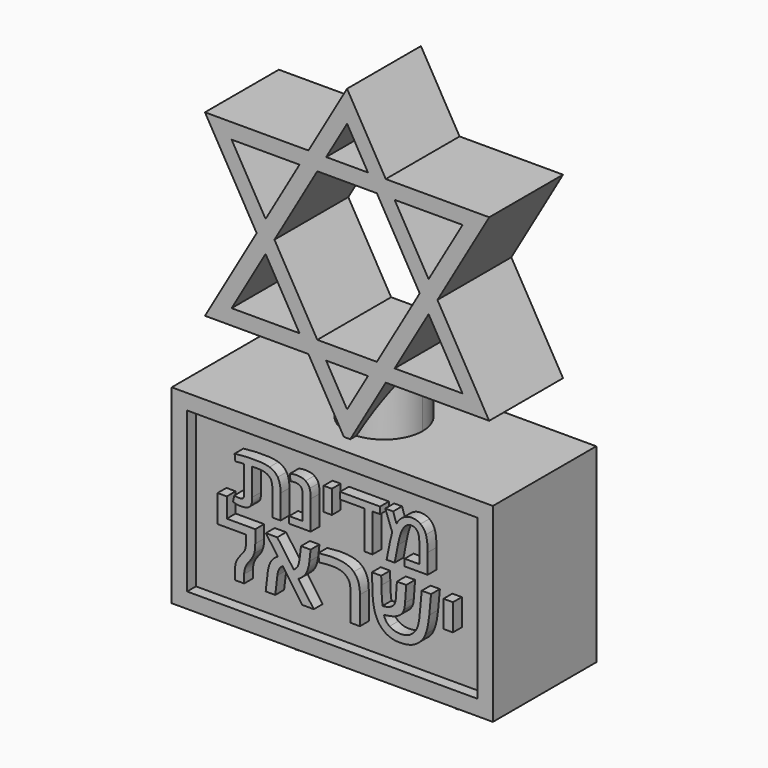
from build123d import *

# Parameters (mm, degrees)
F1_DEPTH  = 15
F9_DEPTH  = 30.9
F10_W     = 47.1880215352
F10_H     = 25.9
F10_W_2   = 1.535165
F10_H_2   = 4.322083
F10_W_3   = 1.333404
F10_H_3   = 3.754038
F11_DEPTH = 1.8
F12_W     = 47.1880215352
F12_H     = 25.9
F12_W_2   = 1.399097
F12_H_2   = 11.579758
F13_DEPTH = 1.8
F14_W     = 1.052821
F14_H     = 3.296269
F14_W_2   = 1.074868
F14_H_2   = 3.026173
F15_DEPTH = 1.8


# Not quite as in the source:
# - ends of sketch curves that miss each other by under 0.0002 mm in the source are joined


with BuildPart() as f1:
    # F0 (on Front) → F1 (new body)
    with BuildSketch(Plane.XZ):
        Polygon((6.283534604, -10.8834011853), (0, 0), (-6.283534604, -10.8834011853), (-23.0940107676, -10.8834011853), (-14.6887726858, -25.4417005926), (-23.0940107676, -40), (-6.283534604, -40), (0, -50.8834011853), (6.2835228852, -40), (23.0940107676, -40), (14.6887589885, -25.4416768682), (23.0939676972, -10.8834011853), align=None)
        Polygon((-2.0189e-06, -45.8833976884), (-3.3967832581, -40), (3.3967728852, -40), align=None, mode=Mode.SUBTRACT)
        Polygon((-18.7638837487, -37.5), (-13.2453970128, -27.9417005926), (-7.726910277, -37.5), align=None, mode=Mode.SUBTRACT)
        Polygon((13.2453846615, -27.9416791995), (18.7638837487, -37.5), (7.7268958663, -37.5), align=None, mode=Mode.SUBTRACT)
        Polygon((-18.7638837487, -13.3834011853), (-11.9086720469, -13.3834011853), (-7.726910277, -13.3834011853), (-13.2453970128, -22.9417005926), align=None, mode=Mode.SUBTRACT)
        Polygon((-4.840158931, -13.3834011853), (4.840158931, -13.3834011853), (11.8020083155, -25.4416780338), (4.8401458663, -37.5), (-4.840158931, -37.5), (-11.8020213399, -25.4417005926), align=None, mode=Mode.SUBTRACT)
        Polygon((11.1853387207, -13.3834011853), (18.7638447161, -13.3834011853), (13.2453826425, -22.9416757026), (7.726910277, -13.3834011853), align=None, mode=Mode.SUBTRACT)
        Polygon((-3.3967832581, -10.8834011853), (0, -5), (3.3967832581, -10.8834011853), (0, -10.8834011853), align=None, mode=Mode.SUBTRACT)
    extrude(amount=F1_DEPTH)

    # F3 (on face) → F4 (join, up to the next surface of F1)
    with BuildSketch(Plane.XY.offset(-50.8834011853)):
        with BuildLine():
            ThreePointArc((0, -1.2164771148), (-4.4431216419, -3.0568783581), (-6.2835228852, -7.5))
            ThreePointArc((-6.2835228852, -7.5), (-4.4431216419, -11.9431216419), (0, -13.7835228852))
            Line((0, -13.7835228852), (0, -1.2164771148))
        make_face()
    extrude(until=Until.NEXT)

    # F3 (on face) → F5 (join, up to the next surface of F1)
    with BuildSketch(Plane.XY.offset(-50.8834011853)):
        with BuildLine():
            ThreePointArc((6.2835228852, -7.5), (4.4431216419, -3.0568783581), (0, -1.2164771148))
            Line((0, -1.2164771148), (0, -13.7835228852))
            ThreePointArc((0, -13.7835228852), (4.4431216419, -11.9431216419), (6.2835228852, -7.5))
        make_face()
    extrude(until=Until.NEXT)

    # F8 (on face) → F9 (join)
    with BuildSketch(Plane.XY.offset(-80.8834011853)):
        Polygon((6.2835228852, 3), (-6.283534604, 3), (-26.0940107676, 3), (-26.0940107676, -18), (-6.283534604, -18), (6.2835228852, -18), (26.0940107676, -18), (26.0940107676, 3), align=None)
    extrude(amount=F9_DEPTH)

    # F10 (on face) → F11 (cut)
    with BuildSketch(Plane.XZ.offset(18)):
        with Locations((0, -65.4334011853)):
            Rectangle(F10_W, F10_H)
        with BuildLine():
            Line((-17.1500309188, -62.6825628694), (-17.1500309188, -65.8709798694))
            Line((-17.1500309188, -65.8709798694), (-12.5209169188, -65.8709798694))
            Line((-12.5209169188, -65.8709798694), (-12.5209169188, -67.9493598694))
            add(Edge.make_bspline(
                [(-12.5209169188, -67.9493598694), (-12.5209169188, -68.5371808694), (-12.5760239188, -69.0147908694), (-12.6862459188, -69.3821818694)],
                knots=[0, 0, 0, 0, 1, 1, 1, 1], degree=3))
            add(Edge.make_bspline(
                [(-12.6862459188, -69.3821818694), (-12.7964619188, -69.7443218694), (-12.9880289188, -70.1117128694), (-13.2609459188, -70.4843478694)],
                knots=[0, 0, 0, 0, 1, 1, 1, 1], degree=3))
            Line((-13.2609459188, -70.4843478694), (-13.6860689188, -71.0511798694))
            add(Edge.make_bspline(
                [(-13.6860689188, -71.0511798694), (-14.1111889188, -71.6232578694), (-14.3237529188, -72.2347008694), (-14.3237529188, -72.8855028694)],
                knots=[0, 0, 0, 0, 1, 1, 1, 1], degree=3))
            Line((-14.3237529188, -72.8855028694), (-14.3237529188, -74.2238538694))
            Line((-14.3237529188, -74.2238538694), (-15.8274269188, -74.2238538694))
            Line((-15.8274269188, -74.2238538694), (-15.8274269188, -73.0980668694))
            add(Edge.make_bspline(
                [(-15.8274269188, -73.0980668694), (-15.8274269188, -72.4210188694), (-15.7618219188, -71.9119208694), (-15.6306079188, -71.5707758694)],
                knots=[0, 0, 0, 0, 1, 1, 1, 1], degree=3))
            add(Edge.make_bspline(
                [(-15.6306079188, -71.5707758694), (-15.4941509188, -71.2296228694), (-15.2973379188, -70.8937248694), (-15.0401629188, -70.5630738694)],
                knots=[0, 0, 0, 0, 1, 1, 1, 1], degree=3))
            Line((-15.0401629188, -70.5630738694), (-14.5678019188, -69.9647538694))
            add(Edge.make_bspline(
                [(-14.5678019188, -69.9647538694), (-14.3368729188, -69.6708448694), (-14.1899169188, -69.4057958694), (-14.1269369188, -69.1696178694)],
                knots=[0, 0, 0, 0, 1, 1, 1, 1], degree=3))
            add(Edge.make_bspline(
                [(-14.1269369188, -69.1696178694), (-14.0587039188, -68.9334378694), (-14.0245919188, -68.6290298694), (-14.0245919188, -68.2563918694)],
                knots=[0, 0, 0, 0, 1, 1, 1, 1], degree=3))
            Line((-14.0245919188, -68.2563918694), (-14.0245919188, -67.1306048694))
            Line((-14.0245919188, -67.1306048694), (-18.6458339188, -67.1306048694))
            Line((-18.6458339188, -67.1306048694), (-18.6458339188, -62.6825628694))
            Line((-18.6458339188, -62.6825628694), (-17.1500309188, -62.6825628694))
        make_face(mode=Mode.SUBTRACT)
        with BuildLine():
            Line((-5.5142679188, -70.6890348694), (-3.0107679188, -74.2238538694))
            Line((-3.0107679188, -74.2238538694), (-4.8687099188, -74.2238538694))
            Line((-4.8687099188, -74.2238538694), (-8.0571299188, -69.7128278694))
            add(Edge.make_bspline(
                [(-8.0571299188, -69.7128278694), (-8.5504799188, -69.9804988694), (-8.8417699188, -70.5210868694), (-8.9309909188, -71.3345958694)],
                knots=[0, 0, 0, 0, 1, 1, 1, 1], degree=3))
            Line((-8.9309909188, -71.3345958694), (-9.2695169188, -74.2238538694))
            Line((-9.2695169188, -74.2238538694), (-10.8282979188, -74.2238538694))
            Line((-10.8282979188, -74.2238538694), (-10.4897749188, -71.3345958694))
            add(Edge.make_bspline(
                [(-10.4897749188, -71.3345958694), (-10.3323209188, -69.9909948694), (-9.7864889188, -69.0830178694), (-8.8522649188, -68.6106598694)],
                knots=[0, 0, 0, 0, 1, 1, 1, 1], degree=3))
            Line((-8.8522649188, -68.6106598694), (-10.7968079188, -65.8709798694))
            Line((-10.7968079188, -65.8709798694), (-8.9467369188, -65.8709798694))
            Line((-8.9467369188, -65.8709798694), (-6.2700389188, -69.6104828694))
            add(Edge.make_bspline(
                [(-6.2700389188, -69.6104828694), (-5.9446369188, -69.3952998694), (-5.7189529188, -69.1538698694), (-5.5929939188, -68.8862018694)],
                knots=[0, 0, 0, 0, 1, 1, 1, 1], degree=3))
            add(Edge.make_bspline(
                [(-5.5929939188, -68.8862018694), (-5.4617799188, -68.6132848694), (-5.3594379188, -68.1671678694), (-5.2859619188, -67.5478568694)],
                knots=[0, 0, 0, 0, 1, 1, 1, 1], degree=3))
            Line((-5.2859619188, -67.5478568694), (-5.0891449188, -65.8709798694))
            Line((-5.0891449188, -65.8709798694), (-3.5303589188, -65.8709798694))
            Line((-3.5303589188, -65.8709798694), (-3.7193039188, -67.5950888694))
            add(Edge.make_bspline(
                [(-3.7193039188, -67.5950888694), (-3.8032789188, -68.3351178694), (-3.9712289188, -68.9439338694), (-4.2231549188, -69.4215438694)],
                knots=[0, 0, 0, 0, 1, 1, 1, 1], degree=3))
            add(Edge.make_bspline(
                [(-4.2231549188, -69.4215438694), (-4.4698309188, -69.8938988694), (-4.9001999188, -70.3163998694), (-5.5142679188, -70.6890348694)],
                knots=[0, 0, 0, 0, 1, 1, 1, 1], degree=3))
        make_face(mode=Mode.SUBTRACT)
        with BuildLine():
            Line((-2.1447749188, -67.2408188694), (-2.2707389188, -65.9497078694))
            add(Edge.make_bspline(
                [(-2.2707389188, -65.9497078694), (-1.4624829188, -65.8342428694), (-0.7198289188, -65.7765058694), (-0.0427829188, -65.7765058694)],
                knots=[0, 0, 0, 0, 1, 1, 1, 1], degree=3))
            add(Edge.make_bspline(
                [(-0.0427829188, -65.7765058694), (1.6472110812, -65.7765058694), (2.8228610812, -66.1045378694), (3.4841620812, -66.7605888694)],
                knots=[0, 0, 0, 0, 1, 1, 1, 1], degree=3))
            add(Edge.make_bspline(
                [(3.4841620812, -66.7605888694), (4.1507110812, -67.4113908694), (4.4839880812, -68.3954738694), (4.4839880812, -69.7128278694)],
                knots=[0, 0, 0, 0, 1, 1, 1, 1], degree=3))
            Line((4.4839880812, -69.7128278694), (4.4839880812, -74.2238538694))
            Line((4.4839880812, -74.2238538694), (2.9881840812, -74.2238538694))
            Line((2.9881840812, -74.2238538694), (2.9881840812, -70.1143348694))
            add(Edge.make_bspline(
                [(2.9881840812, -70.1143348694), (2.9881840812, -69.3533108694), (2.9068340812, -68.7786138694), (2.7441360812, -68.3902248694)],
                knots=[0, 0, 0, 0, 1, 1, 1, 1], degree=3))
            add(Edge.make_bspline(
                [(2.7441360812, -68.3902248694), (2.5814320812, -68.0018448694), (2.2691500812, -67.6869378694), (1.8072900812, -67.4455088694)],
                knots=[0, 0, 0, 0, 1, 1, 1, 1], degree=3))
            add(Edge.make_bspline(
                [(1.8072900812, -67.4455088694), (1.3454280812, -67.2040838694), (0.6998730812, -67.0833668694), (-0.1293809188, -67.0833668694)],
                knots=[0, 0, 0, 0, 1, 1, 1, 1], degree=3))
            add(Edge.make_bspline(
                [(-0.1293809188, -67.0833668694), (-0.6909599188, -67.0833668694), (-1.3627589188, -67.1358538694), (-2.1447749188, -67.2408188694)],
                knots=[0, 0, 0, 0, 1, 1, 1, 1], degree=3))
        make_face(mode=Mode.SUBTRACT)
        with BuildLine():
            Line((6.4206590812, -65.8709798694), (7.9479490812, -65.8709798694))
            Line((7.9479490812, -65.8709798694), (7.9794420812, -67.2250728694))
            add(Edge.make_bspline(
                [(7.9794420812, -67.2250728694), (8.0109330812, -68.6159098694), (8.0712890812, -69.5789958694), (8.1605130812, -70.1143348694)],
                knots=[0, 0, 0, 0, 1, 1, 1, 1], degree=3))
            add(Edge.make_bspline(
                [(8.1605130812, -70.1143348694), (8.7168440812, -70.1143348694), (9.2180680812, -69.9752498694), (9.6641850812, -69.6970858694)],
                knots=[0, 0, 0, 0, 1, 1, 1, 1], degree=3))
            add(Edge.make_bspline(
                [(9.6641850812, -69.6970858694), (10.1103020812, -69.4189158694), (10.3333620812, -68.8914488694), (10.3333620812, -68.1146858694)],
                knots=[0, 0, 0, 0, 1, 1, 1, 1], degree=3))
            Line((10.3333620812, -68.1146858694), (10.4986850812, -65.8709798694))
            Line((10.4986850812, -65.8709798694), (12.0102310812, -65.8709798694))
            Line((12.0102310812, -65.8709798694), (11.8212880812, -68.5004438694))
            add(Edge.make_bspline(
                [(11.8212880812, -68.5004438694), (11.7897980812, -68.9465608694), (11.7399380812, -69.2850838694), (11.6717080812, -69.5160118694)],
                knots=[0, 0, 0, 0, 1, 1, 1, 1], degree=3))
            add(Edge.make_bspline(
                [(11.6717080812, -69.5160118694), (11.6034810812, -69.7469458694), (11.4617710812, -69.9909948694), (11.2465850812, -70.2481698694)],
                knots=[0, 0, 0, 0, 1, 1, 1, 1], degree=3))
            add(Edge.make_bspline(
                [(11.2465850812, -70.2481698694), (11.0366460812, -70.5053418694), (10.7007500812, -70.7310238694), (10.2388880812, -70.9252178694)],
                knots=[0, 0, 0, 0, 1, 1, 1, 1], degree=3))
            add(Edge.make_bspline(
                [(10.2388880812, -70.9252178694), (9.7822750812, -71.1141598694), (9.1655830812, -71.2401218694), (8.3888170812, -71.3031028694)],
                knots=[0, 0, 0, 0, 1, 1, 1, 1], degree=3))
            add(Edge.make_bspline(
                [(8.3888170812, -71.3031028694), (8.5200310812, -71.8699348694), (8.8244380812, -72.3239228694), (9.3020460812, -72.6650698694)],
                knots=[0, 0, 0, 0, 1, 1, 1, 1], degree=3))
            add(Edge.make_bspline(
                [(9.3020460812, -72.6650698694), (9.7796530812, -73.0062178694), (10.3674770812, -73.1767928694), (11.0655170812, -73.1767928694)],
                knots=[0, 0, 0, 0, 1, 1, 1, 1], degree=3))
            add(Edge.make_bspline(
                [(11.0655170812, -73.1767928694), (11.7110690812, -73.1767928694), (12.2647810812, -73.0245898694), (12.7266430812, -72.7201798694)],
                knots=[0, 0, 0, 0, 1, 1, 1, 1], degree=3))
            add(Edge.make_bspline(
                [(12.7266430812, -72.7201798694), (13.1885030812, -72.4105198694), (13.5296530812, -72.0142628694), (13.7500880812, -71.5314088694)],
                knots=[0, 0, 0, 0, 1, 1, 1, 1], degree=3))
            add(Edge.make_bspline(
                [(13.7500880812, -71.5314088694), (13.9705210812, -71.0433028694), (14.1174770812, -70.3505148694), (14.1909560812, -69.4530318694)],
                knots=[0, 0, 0, 0, 1, 1, 1, 1], degree=3))
            Line((14.1909560812, -69.4530318694), (14.5294760812, -65.8709798694))
            Line((14.5294760812, -65.8709798694), (16.0410270812, -65.8709798694))
            Line((16.0410270812, -65.8709798694), (15.7576110812, -68.9649308694))
            add(Edge.make_bspline(
                [(15.7576110812, -68.9649308694), (15.6473920812, -70.1248298694), (15.4505760812, -71.0905408694), (15.1671630812, -71.8620608694)],
                knots=[0, 0, 0, 0, 1, 1, 1, 1], degree=3))
            add(Edge.make_bspline(
                [(15.1671630812, -71.8620608694), (14.8837470812, -72.6335798694), (14.3903970812, -73.2581428694), (13.6871080812, -73.7357478694)],
                knots=[0, 0, 0, 0, 1, 1, 1, 1], degree=3))
            add(Edge.make_bspline(
                [(13.6871080812, -73.7357478694), (12.9890650812, -74.2133558694), (12.0863370812, -74.4521608694), (10.9789170812, -74.4521608694)],
                knots=[0, 0, 0, 0, 1, 1, 1, 1], degree=3))
            add(Edge.make_bspline(
                [(10.9789170812, -74.4521608694), (9.9974610812, -74.4521608694), (9.1734570812, -74.2159798694), (8.5069070812, -73.7436248694)],
                knots=[0, 0, 0, 0, 1, 1, 1, 1], degree=3))
            add(Edge.make_bspline(
                [(8.5069070812, -73.7436248694), (7.8456070812, -73.2660168694), (7.3496270812, -72.5863438694), (7.0189780812, -71.7046088694)],
                knots=[0, 0, 0, 0, 1, 1, 1, 1], degree=3))
            add(Edge.make_bspline(
                [(7.0189780812, -71.7046088694), (6.6935760812, -70.8228698694), (6.5308750812, -69.6472258694), (6.5308750812, -68.1776638694)],
                knots=[0, 0, 0, 0, 1, 1, 1, 1], degree=3))
            Line((6.5308750812, -68.1776638694), (6.4206590812, -65.8709798694))
        make_face(mode=Mode.SUBTRACT)
        with Locations((18.8318745812, -68.0320213694)):
            Rectangle(F10_W_2, F10_H_2, mode=Mode.SUBTRACT)
        with BuildLine():
            add(Edge.make_bspline(
                [(-14.8649959188, -63.3475318694), (-15.2935109188, -63.3475318694), (-15.7197419188, -63.2723138694), (-16.1436969188, -63.1218778694)],
                knots=[0, 0, 0, 0, 1, 1, 1, 1], degree=3))
            Line((-16.1436969188, -63.1218778694), (-15.9180429188, -62.1440398694))
            add(Edge.make_bspline(
                [(-15.9180429188, -62.1440398694), (-15.6809959188, -62.2260938694), (-15.4234319188, -62.2671228694), (-15.1453549188, -62.2671228694)],
                knots=[0, 0, 0, 0, 1, 1, 1, 1], degree=3))
            add(Edge.make_bspline(
                [(-15.1453549188, -62.2671228694), (-14.8308099188, -62.2671228694), (-14.6142719188, -62.1987438694), (-14.4957479188, -62.0619838694)],
                knots=[0, 0, 0, 0, 1, 1, 1, 1], degree=3))
            add(Edge.make_bspline(
                [(-14.4957479188, -62.0619838694), (-14.3772249188, -61.9206638694), (-14.3179619188, -61.6676628694), (-14.3179619188, -61.3029698694)],
                knots=[0, 0, 0, 0, 1, 1, 1, 1], degree=3))
            Line((-14.3179619188, -61.3029698694), (-14.3179619188, -57.1181368694))
            add(Edge.make_bspline(
                [(-14.3179619188, -57.1181368694), (-14.7100049188, -57.1181368694), (-15.1909429188, -57.1591628694), (-15.7607689188, -57.2412198694)],
                knots=[0, 0, 0, 0, 1, 1, 1, 1], degree=3))
            Line((-15.7607689188, -57.2412198694), (-15.8770159188, -56.1539808694))
            add(Edge.make_bspline(
                [(-15.8770159188, -56.1539808694), (-14.8376459188, -56.0217818694), (-13.7823209188, -55.9556828694), (-12.7110419188, -55.9556828694)],
                knots=[0, 0, 0, 0, 1, 1, 1, 1], degree=3))
            add(Edge.make_bspline(
                [(-12.7110419188, -55.9556828694), (-11.6260869188, -55.9556828694), (-10.7918519188, -56.0468578694), (-10.2083459188, -56.2292018694)],
                knots=[0, 0, 0, 0, 1, 1, 1, 1], degree=3))
            add(Edge.make_bspline(
                [(-10.2083459188, -56.2292018694), (-9.6248399188, -56.4115478694), (-9.1803709188, -56.7466078694), (-8.8749449188, -57.2343808694)],
                knots=[0, 0, 0, 0, 1, 1, 1, 1], degree=3))
            add(Edge.make_bspline(
                [(-8.8749449188, -57.2343808694), (-8.5649549188, -57.7175988694), (-8.4099609188, -58.4310258694), (-8.4099609188, -59.3746638694)],
                knots=[0, 0, 0, 0, 1, 1, 1, 1], degree=3))
            Line((-8.4099609188, -59.3746638694), (-8.4099609188, -63.2928168694))
            Line((-8.4099609188, -63.2928168694), (-9.7160119188, -63.2928168694))
            Line((-9.7160119188, -63.2928168694), (-9.7160119188, -59.7234028694))
            add(Edge.make_bspline(
                [(-9.7160119188, -59.7234028694), (-9.7160119188, -59.0168088694), (-9.7707149188, -58.4994058694), (-9.8801219188, -58.1711808694)],
                knots=[0, 0, 0, 0, 1, 1, 1, 1], degree=3))
            add(Edge.make_bspline(
                [(-9.8801219188, -58.1711808694), (-9.9849729188, -57.8429618694), (-10.2174649188, -57.5762788694), (-10.5775939188, -57.3711428694)],
                knots=[0, 0, 0, 0, 1, 1, 1, 1], degree=3))
            add(Edge.make_bspline(
                [(-10.5775939188, -57.3711428694), (-10.9377299188, -57.1660038694), (-11.5326319188, -57.0634338694), (-12.3623029188, -57.0634338694)],
                knots=[0, 0, 0, 0, 1, 1, 1, 1], degree=3))
            Line((-12.3623029188, -57.0634338694), (-13.0187459188, -57.0771208694))
            Line((-13.0187459188, -57.0771208694), (-13.0187459188, -61.4739288694))
            add(Edge.make_bspline(
                [(-13.0187459188, -61.4739288694), (-13.0187459188, -61.9297968694), (-13.0620559188, -62.2785308694), (-13.1486699188, -62.5201378694)],
                knots=[0, 0, 0, 0, 1, 1, 1, 1], degree=3))
            add(Edge.make_bspline(
                [(-13.1486699188, -62.5201378694), (-13.2307259188, -62.7617458694), (-13.4062309188, -62.9600458694), (-13.6751919188, -63.1150398694)],
                knots=[0, 0, 0, 0, 1, 1, 1, 1], degree=3))
            add(Edge.make_bspline(
                [(-13.6751919188, -63.1150398694), (-13.9395949188, -63.2700338694), (-14.3361959188, -63.3475318694), (-14.8649959188, -63.3475318694)],
                knots=[0, 0, 0, 0, 1, 1, 1, 1], degree=3))
        make_face(mode=Mode.SUBTRACT)
        with BuildLine():
            Line((-3.5071429188, -58.6019738694), (-3.5071429188, -63.2928168694))
            Line((-3.5071429188, -63.2928168694), (-7.0081799188, -63.2928168694))
            Line((-7.0081799188, -63.2928168694), (-7.0081799188, -62.1987438694))
            Line((-7.0081799188, -62.1987438694), (-4.8131909188, -62.1987438694))
            Line((-4.8131909188, -62.1987438694), (-4.8131909188, -58.6430028694))
            add(Edge.make_bspline(
                [(-4.8131909188, -58.6430028694), (-4.8131909188, -58.2509598694), (-4.8428249188, -57.9546458694), (-4.9020889188, -57.7540678694)],
                knots=[0, 0, 0, 0, 1, 1, 1, 1], degree=3))
            add(Edge.make_bspline(
                [(-4.9020889188, -57.7540678694), (-4.9613499188, -57.5489258694), (-5.0889929188, -57.3848198694), (-5.2850099188, -57.2617338694)],
                knots=[0, 0, 0, 0, 1, 1, 1, 1], degree=3))
            add(Edge.make_bspline(
                [(-5.2850099188, -57.2617338694), (-5.4764759188, -57.1386508694), (-5.7340399188, -57.0771098694), (-6.0577039188, -57.0771098694)],
                knots=[0, 0, 0, 0, 1, 1, 1, 1], degree=3))
            add(Edge.make_bspline(
                [(-6.0577039188, -57.0771098694), (-6.3357799188, -57.0771098694), (-6.5842259188, -57.0999138694), (-6.8030389188, -57.1454898694)],
                knots=[0, 0, 0, 0, 1, 1, 1, 1], degree=3))
            Line((-6.8030389188, -57.1454898694), (-6.8987709188, -56.1061188694))
            add(Edge.make_bspline(
                [(-6.8987709188, -56.1061188694), (-6.5933419188, -56.0058278694), (-6.2195359188, -55.9556828694), (-5.7773439188, -55.9556828694)],
                knots=[0, 0, 0, 0, 1, 1, 1, 1], degree=3))
            add(Edge.make_bspline(
                [(-5.7773439188, -55.9556828694), (-5.1573699188, -55.9556828694), (-4.6832729188, -56.0719278694), (-4.3550489188, -56.3044198694)],
                knots=[0, 0, 0, 0, 1, 1, 1, 1], degree=3))
            add(Edge.make_bspline(
                [(-4.3550489188, -56.3044198694), (-4.0268239188, -56.5369088694), (-3.8034569188, -56.8241058694), (-3.6849289188, -57.1660038694)],
                knots=[0, 0, 0, 0, 1, 1, 1, 1], degree=3))
            add(Edge.make_bspline(
                [(-3.6849289188, -57.1660038694), (-3.5664039188, -57.5033448694), (-3.5071429188, -57.9819988694), (-3.5071429188, -58.6019738694)],
                knots=[0, 0, 0, 0, 1, 1, 1, 1], degree=3))
        make_face(mode=Mode.SUBTRACT)
        with Locations((-0.7411849188, -57.9147578694)):
            Rectangle(F10_W_3, F10_H_3, mode=Mode.SUBTRACT)
        Polygon((7.7618240812, -56.0377388694), (7.7618240812, -57.1318128694), (6.5241490812, -57.1318128694), (6.5241490812, -63.2928168694), (5.2249370812, -63.2928168694), (5.2249370812, -57.1318128694), (1.2589190812, -57.1318128694), (1.2589190812, -56.0377388694), align=None, mode=Mode.SUBTRACT)
        with BuildLine():
            add(Edge.make_bspline(
                [(9.3960960812, -60.4618998694), (9.4508000812, -60.1929418694), (9.5624830812, -59.7279588694), (9.7311560812, -59.0669568694)],
                knots=[0, 0, 0, 0, 1, 1, 1, 1], degree=3))
            Line((9.7311560812, -59.0669568694), (8.6097290812, -56.0377388694))
            Line((8.6097290812, -56.0377388694), (9.8884270812, -56.0377388694))
            Line((9.8884270812, -56.0377388694), (10.4217880812, -57.6378208694))
            add(Edge.make_bspline(
                [(10.4217880812, -57.6378208694), (10.6360450812, -57.1682788694), (10.9711050812, -56.7716808694), (11.4269700812, -56.4480168694)],
                knots=[0, 0, 0, 0, 1, 1, 1, 1], degree=3))
            add(Edge.make_bspline(
                [(11.4269700812, -56.4480168694), (11.8828350812, -56.1197928694), (12.3728890812, -55.9556828694), (12.8971310812, -55.9556828694)],
                knots=[0, 0, 0, 0, 1, 1, 1, 1], degree=3))
            add(Edge.make_bspline(
                [(12.8971310812, -55.9556828694), (13.4532860812, -55.9556828694), (13.9319440812, -56.0992808694), (14.3331060812, -56.3864758694)],
                knots=[0, 0, 0, 0, 1, 1, 1, 1], degree=3))
            add(Edge.make_bspline(
                [(14.3331060812, -56.3864758694), (14.7388260812, -56.6691098694), (15.0328560812, -57.0839478694), (15.2152030812, -57.6309828694)],
                knots=[0, 0, 0, 0, 1, 1, 1, 1], degree=3))
            add(Edge.make_bspline(
                [(15.2152030812, -57.6309828694), (15.3975460812, -58.1780218694), (15.4887210812, -59.0008548694), (15.4887210812, -60.0994868694)],
                knots=[0, 0, 0, 0, 1, 1, 1, 1], degree=3))
            Line((15.4887210812, -60.0994868694), (15.4887210812, -63.2928168694))
            Line((15.4887210812, -63.2928168694), (11.7483540812, -63.2928168694))
            Line((11.7483540812, -63.2928168694), (11.7483540812, -62.1987438694))
            Line((11.7483540812, -62.1987438694), (14.1689930812, -62.1987438694))
            Line((14.1689930812, -62.1987438694), (14.1689930812, -60.0721398694))
            add(Edge.make_bspline(
                [(14.1689930812, -60.0721398694), (14.1689930812, -59.2698158694), (14.1416460812, -58.6863068694), (14.0869370812, -58.3216198694)],
                knots=[0, 0, 0, 0, 1, 1, 1, 1], degree=3))
            add(Edge.make_bspline(
                [(14.0869370812, -58.3216198694), (14.0367920812, -57.9523688694), (13.9023100812, -57.6537748694), (13.6834950812, -57.4258438694)],
                knots=[0, 0, 0, 0, 1, 1, 1, 1], degree=3))
            add(Edge.make_bspline(
                [(13.6834950812, -57.4258438694), (13.4692400812, -57.1933548694), (13.1980020812, -57.0771098694), (12.8697810812, -57.0771098694)],
                knots=[0, 0, 0, 0, 1, 1, 1, 1], degree=3))
            add(Edge.make_bspline(
                [(12.8697810812, -57.0771098694), (12.3592100812, -57.0771098694), (11.9238620812, -57.3415098694), (11.5637270812, -57.8703128694)],
                knots=[0, 0, 0, 0, 1, 1, 1, 1], degree=3))
            add(Edge.make_bspline(
                [(11.5637270812, -57.8703128694), (11.2081550812, -58.3945568694), (10.9050030812, -59.3062848694), (10.6542800812, -60.6054968694)],
                knots=[0, 0, 0, 0, 1, 1, 1, 1], degree=3))
            Line((10.6542800812, -60.6054968694), (10.1414310812, -63.2928168694))
            Line((10.1414310812, -63.2928168694), (8.8217060812, -63.2928168694))
            Line((8.8217060812, -63.2928168694), (9.3960960812, -60.4618998694))
        make_face(mode=Mode.SUBTRACT)
    extrude(amount=-F11_DEPTH, mode=Mode.SUBTRACT)

    # F12 (on face) → F13 (cut)
    with BuildSketch(Plane(origin=(0, 3, 0), x_dir=(-1, 0, 0), z_dir=(0, 1, 0))):
        with Locations((0, -65.4334011853)):
            Rectangle(F12_W, F12_H)
        Polygon((-16.4047140732, -75.173243564), (-16.4047140732, -76.304426564), (-20.7806120732, -76.304426564), (-20.7806120732, -75.173243564), (-19.3294260732, -75.173243564), (-19.3294260732, -66.354464564), (-20.7806120732, -66.354464564), (-20.7806120732, -65.223275564), (-16.4047140732, -65.223275564), (-16.4047140732, -66.354464564), (-17.8559010732, -66.354464564), (-17.8559010732, -75.173243564), align=None, mode=Mode.SUBTRACT)
        with BuildLine():
            add(Edge.make_bspline(
                [(-8.5831630732, -72.449465564), (-8.2309120732, -72.816605564), (-8.0547860732, -73.302816564), (-8.0547860732, -73.908100564)],
                knots=[0, 0, 0, 0, 1, 1, 1, 1], degree=3))
            add(Edge.make_bspline(
                [(-8.0547860732, -73.908100564), (-8.0547860732, -74.667184564), (-8.3698290732, -75.289831564), (-8.9999150732, -75.776041564)],
                knots=[0, 0, 0, 0, 1, 1, 1, 1], degree=3))
            add(Edge.make_bspline(
                [(-8.9999150732, -75.776041564), (-9.6250440732, -76.262252564), (-10.4808770732, -76.505357564), (-11.5674110732, -76.505357564)],
                knots=[0, 0, 0, 0, 1, 1, 1, 1], degree=3))
            add(Edge.make_bspline(
                [(-11.5674110732, -76.505357564), (-12.1826160732, -76.505357564), (-12.7482090732, -76.433418564), (-13.2641880732, -76.289539564)],
                knots=[0, 0, 0, 0, 1, 1, 1, 1], degree=3))
            add(Edge.make_bspline(
                [(-13.2641880732, -76.289539564), (-13.7752060732, -76.140701564), (-14.2043620732, -75.979459564), (-14.5516570732, -75.805813564)],
                knots=[0, 0, 0, 0, 1, 1, 1, 1], degree=3))
            Line((-14.5516570732, -75.805813564), (-14.5516570732, -74.235543564))
            Line((-14.5516570732, -74.235543564), (-14.4772300732, -74.235543564))
            add(Edge.make_bspline(
                [(-14.4772300732, -74.235543564), (-14.0356720732, -74.567957564), (-13.5445010732, -74.833390564), (-13.0037170732, -75.031841564)],
                knots=[0, 0, 0, 0, 1, 1, 1, 1], degree=3))
            add(Edge.make_bspline(
                [(-13.0037170732, -75.031841564), (-12.4629300732, -75.225335564), (-11.9444710732, -75.322081564), (-11.4483390732, -75.322081564)],
                knots=[0, 0, 0, 0, 1, 1, 1, 1], degree=3))
            add(Edge.make_bspline(
                [(-11.4483390732, -75.322081564), (-10.8331320732, -75.322081564), (-10.3518820732, -75.222855564), (-10.0045890732, -75.024402564)],
                knots=[0, 0, 0, 0, 1, 1, 1, 1], degree=3))
            add(Edge.make_bspline(
                [(-10.0045890732, -75.024402564), (-9.6572980732, -74.825947564), (-9.4836520732, -74.513382564), (-9.4836520732, -74.086707564)],
                knots=[0, 0, 0, 0, 1, 1, 1, 1], degree=3))
            add(Edge.make_bspline(
                [(-9.4836520732, -74.086707564), (-9.4836520732, -73.759260564), (-9.5779160732, -73.511193564), (-9.7664440732, -73.342507564)],
                knots=[0, 0, 0, 0, 1, 1, 1, 1], degree=3))
            add(Edge.make_bspline(
                [(-9.7664440732, -73.342507564), (-9.9549760732, -73.173821564), (-10.3171560732, -73.029941564), (-10.8529830732, -72.910868564)],
                knots=[0, 0, 0, 0, 1, 1, 1, 1], degree=3))
            add(Edge.make_bspline(
                [(-10.8529830732, -72.910868564), (-11.0514340732, -72.866218564), (-11.3119030732, -72.814125564), (-11.6343910732, -72.754587564)],
                knots=[0, 0, 0, 0, 1, 1, 1, 1], degree=3))
            add(Edge.make_bspline(
                [(-11.6343910732, -72.754587564), (-11.9519160732, -72.695051564), (-12.2421540732, -72.630553564), (-12.5051060732, -72.561093564)],
                knots=[0, 0, 0, 0, 1, 1, 1, 1], degree=3))
            add(Edge.make_bspline(
                [(-12.5051060732, -72.561093564), (-13.2344230732, -72.367603564), (-13.7528800732, -72.084808564), (-14.0604780732, -71.712707564)],
                knots=[0, 0, 0, 0, 1, 1, 1, 1], degree=3))
            add(Edge.make_bspline(
                [(-14.0604780732, -71.712707564), (-14.3631240732, -71.335645564), (-14.5144460732, -70.874242564), (-14.5144460732, -70.328498564)],
                knots=[0, 0, 0, 0, 1, 1, 1, 1], degree=3))
            add(Edge.make_bspline(
                [(-14.5144460732, -70.328498564), (-14.5144460732, -69.986162564), (-14.4449880732, -69.663673564), (-14.3060700732, -69.361031564)],
                knots=[0, 0, 0, 0, 1, 1, 1, 1], degree=3))
            add(Edge.make_bspline(
                [(-14.3060700732, -69.361031564), (-14.1621920732, -69.058391564), (-13.9463730732, -68.787999564), (-13.6586130732, -68.549854564)],
                knots=[0, 0, 0, 0, 1, 1, 1, 1], degree=3))
            add(Edge.make_bspline(
                [(-13.6586130732, -68.549854564), (-13.3807790732, -68.316673564), (-13.0285250732, -68.133104564), (-12.6018520732, -67.999148564)],
                knots=[0, 0, 0, 0, 1, 1, 1, 1], degree=3))
            add(Edge.make_bspline(
                [(-12.6018520732, -67.999148564), (-12.1702140732, -67.860231564), (-11.6889650732, -67.790772564), (-11.1581050732, -67.790772564)],
                knots=[0, 0, 0, 0, 1, 1, 1, 1], degree=3))
            add(Edge.make_bspline(
                [(-11.1581050732, -67.790772564), (-10.6619690732, -67.790772564), (-10.1608710732, -67.852788564), (-9.6548110732, -67.976819564)],
                knots=[0, 0, 0, 0, 1, 1, 1, 1], degree=3))
            add(Edge.make_bspline(
                [(-9.6548110732, -67.976819564), (-9.1437970732, -68.095890564), (-8.7196050732, -68.242251564), (-8.3822340732, -68.415900564)],
                knots=[0, 0, 0, 0, 1, 1, 1, 1], degree=3))
            Line((-8.3822340732, -68.415900564), (-8.3822340732, -69.911743564))
            Line((-8.3822340732, -69.911743564), (-8.4566510732, -69.911743564))
            add(Edge.make_bspline(
                [(-8.4566510732, -69.911743564), (-8.8138670732, -69.648793564), (-9.2479850732, -69.428013564), (-9.7590050732, -69.249404564)],
                knots=[0, 0, 0, 0, 1, 1, 1, 1], degree=3))
            add(Edge.make_bspline(
                [(-9.7590050732, -69.249404564), (-10.2700210732, -69.065834564), (-10.7711150732, -68.974048564), (-11.2622870732, -68.974048564)],
                knots=[0, 0, 0, 0, 1, 1, 1, 1], degree=3))
            add(Edge.make_bspline(
                [(-11.2622870732, -68.974048564), (-11.7733050732, -68.974048564), (-12.2049410732, -69.073276564), (-12.5571960732, -69.271731564)],
                knots=[0, 0, 0, 0, 1, 1, 1, 1], degree=3))
            add(Edge.make_bspline(
                [(-12.5571960732, -69.271731564), (-12.9094520732, -69.465222564), (-13.0855810732, -69.755461564), (-13.0855810732, -70.142448564)],
                knots=[0, 0, 0, 0, 1, 1, 1, 1], degree=3))
            add(Edge.make_bspline(
                [(-13.0855810732, -70.142448564), (-13.0855810732, -70.484778564), (-12.9789120732, -70.742768564), (-12.7655750732, -70.916417564)],
                knots=[0, 0, 0, 0, 1, 1, 1, 1], degree=3))
            add(Edge.make_bspline(
                [(-12.7655750732, -70.916417564), (-12.5571970732, -71.090061564), (-12.2198260732, -71.231458564), (-11.7534640732, -71.340609564)],
                knots=[0, 0, 0, 0, 1, 1, 1, 1], degree=3))
            add(Edge.make_bspline(
                [(-11.7534640732, -71.340609564), (-11.4954730732, -71.400144564), (-11.2077140732, -71.459681564), (-10.8901880732, -71.519219564)],
                knots=[0, 0, 0, 0, 1, 1, 1, 1], degree=3))
            add(Edge.make_bspline(
                [(-10.8901880732, -71.519219564), (-10.5677000732, -71.578752564), (-10.2997890732, -71.633326564), (-10.0864530732, -71.682939564)],
                knots=[0, 0, 0, 0, 1, 1, 1, 1], degree=3))
            add(Edge.make_bspline(
                [(-10.0864530732, -71.682939564), (-9.4365160732, -71.831779564), (-8.9354190732, -72.087288564), (-8.5831630732, -72.449465564)],
                knots=[0, 0, 0, 0, 1, 1, 1, 1], degree=3))
        make_face(mode=Mode.SUBTRACT)
        with BuildLine():
            Line((-0.8583680732, -68.081013564), (-0.8583680732, -69.517320564))
            Line((-0.8583680732, -69.517320564), (-0.9327870732, -69.517318564))
            add(Edge.make_bspline(
                [(-0.9327870732, -69.517318564), (-1.1411610732, -69.467703564), (-1.3445750732, -69.432972564), (-1.5430280732, -69.413124564)],
                knots=[0, 0, 0, 0, 1, 1, 1, 1], degree=3))
            add(Edge.make_bspline(
                [(-1.5430280732, -69.413124564), (-1.7365210732, -69.388307564), (-1.9672250732, -69.375899564), (-2.2351380732, -69.375899564)],
                knots=[0, 0, 0, 0, 1, 1, 1, 1], degree=3))
            add(Edge.make_bspline(
                [(-2.2351380732, -69.375899564), (-2.6667740732, -69.375899564), (-3.0835250732, -69.472646564), (-3.4853910732, -69.666139564)],
                knots=[0, 0, 0, 0, 1, 1, 1, 1], degree=3))
            add(Edge.make_bspline(
                [(-3.4853910732, -69.666139564), (-3.8872590732, -69.854667564), (-4.2742430732, -70.100252564), (-4.6463430732, -70.402894564)],
                knots=[0, 0, 0, 0, 1, 1, 1, 1], degree=3))
            Line((-4.6463430732, -70.402894564), (-4.6463430732, -76.304404564))
            Line((-4.6463430732, -76.304404564), (-6.0454430732, -76.304404564))
            Line((-6.0454430732, -76.304404564), (-6.0454430732, -67.991684564))
            Line((-6.0454430732, -67.991684564), (-4.6463430732, -67.991684564))
            Line((-4.6463430732, -67.991684564), (-4.6463430732, -69.219618564))
            add(Edge.make_bspline(
                [(-4.6463430732, -69.219618564), (-4.0906760732, -68.773096564), (-3.6019850732, -68.458049564), (-3.1802690732, -68.274479564)],
                knots=[0, 0, 0, 0, 1, 1, 1, 1], degree=3))
            add(Edge.make_bspline(
                [(-3.1802690732, -68.274479564), (-2.7535960732, -68.085949564), (-2.3194800732, -67.991684564), (-1.8779210732, -67.991684564)],
                knots=[0, 0, 0, 0, 1, 1, 1, 1], degree=3))
            add(Edge.make_bspline(
                [(-1.8779210732, -67.991684564), (-1.6348150732, -67.991684564), (-1.4586870732, -67.999134564), (-1.3495390732, -68.014036564)],
                knots=[0, 0, 0, 0, 1, 1, 1, 1], degree=3))
            add(Edge.make_bspline(
                [(-1.3495390732, -68.014036564), (-1.2403890732, -68.023989564), (-1.0766650732, -68.046314564), (-0.8583680732, -68.081013564)],
                knots=[0, 0, 0, 0, 1, 1, 1, 1], degree=3))
        make_face(mode=Mode.SUBTRACT)
        with BuildLine():
            Line((6.6655019268, -70.663383564), (6.6655019268, -76.304426564))
            Line((6.6655019268, -76.304426564), (5.2738469268, -76.304426564))
            Line((5.2738469268, -76.304426564), (5.2738469268, -75.418824564))
            add(Edge.make_bspline(
                [(5.2738469268, -75.418824564), (5.1498139268, -75.503165564), (4.9811289268, -75.622238564), (4.7677909268, -75.776041564)],
                knots=[0, 0, 0, 0, 1, 1, 1, 1], degree=3))
            add(Edge.make_bspline(
                [(4.7677909268, -75.776041564), (4.5594149268, -75.924882564), (4.3560009268, -76.043954564), (4.1575479268, -76.133258564)],
                knots=[0, 0, 0, 0, 1, 1, 1, 1], degree=3))
            add(Edge.make_bspline(
                [(4.1575479268, -76.133258564), (3.9243649268, -76.247370564), (3.6564509268, -76.341635564), (3.3538069268, -76.416054564)],
                knots=[0, 0, 0, 0, 1, 1, 1, 1], degree=3))
            add(Edge.make_bspline(
                [(3.3538069268, -76.416054564), (3.0511669268, -76.495435564), (2.6964319268, -76.535126564), (2.2896009268, -76.535126564)],
                knots=[0, 0, 0, 0, 1, 1, 1, 1], degree=3))
            add(Edge.make_bspline(
                [(2.2896009268, -76.535126564), (1.5404379268, -76.535126564), (0.9053869268, -76.287058564), (0.3844489268, -75.790923564)],
                knots=[0, 0, 0, 0, 1, 1, 1, 1], degree=3))
            add(Edge.make_bspline(
                [(0.3844489268, -75.790923564), (-0.1364920732, -75.294791564), (-0.3969630732, -74.662223564), (-0.3969630732, -73.893218564)],
                knots=[0, 0, 0, 0, 1, 1, 1, 1], degree=3))
            add(Edge.make_bspline(
                [(-0.3969630732, -73.893218564), (-0.3969630732, -73.263125564), (-0.2630070732, -72.754587564), (0.0049049268, -72.367604564)],
                knots=[0, 0, 0, 0, 1, 1, 1, 1], degree=3))
            add(Edge.make_bspline(
                [(0.0049049268, -72.367604564), (0.2777799268, -71.975658564), (0.6647639268, -71.668053564), (1.1658569268, -71.444791564)],
                knots=[0, 0, 0, 0, 1, 1, 1, 1], degree=3))
            add(Edge.make_bspline(
                [(1.1658569268, -71.444791564), (1.6719149268, -71.221534564), (2.2796809268, -71.070215564), (2.9891539268, -70.990834564)],
                knots=[0, 0, 0, 0, 1, 1, 1, 1], degree=3))
            add(Edge.make_bspline(
                [(2.9891539268, -70.990834564), (3.6986249268, -70.911452564), (4.4601889268, -70.851915564), (5.2738469268, -70.812224564)],
                knots=[0, 0, 0, 0, 1, 1, 1, 1], degree=3))
            Line((5.2738469268, -70.812224564), (5.2738469268, -70.596406564))
            add(Edge.make_bspline(
                [(5.2738469268, -70.596406564), (5.2738469268, -70.278881564), (5.2167909268, -70.015930564), (5.1026789268, -69.807552564)],
                knots=[0, 0, 0, 0, 1, 1, 1, 1], degree=3))
            add(Edge.make_bspline(
                [(5.1026789268, -69.807552564), (4.9935309268, -69.599178564), (4.8347679268, -69.435454564), (4.6263919268, -69.316381564)],
                knots=[0, 0, 0, 0, 1, 1, 1, 1], degree=3))
            add(Edge.make_bspline(
                [(4.6263919268, -69.316381564), (4.4279389268, -69.202271564), (4.1897949268, -69.125370564), (3.9119579268, -69.085678564)],
                knots=[0, 0, 0, 0, 1, 1, 1, 1], degree=3))
            add(Edge.make_bspline(
                [(3.9119579268, -69.085678564), (3.6341239268, -69.045989564), (3.3438859268, -69.026144564), (3.0412459268, -69.026144564)],
                knots=[0, 0, 0, 0, 1, 1, 1, 1], degree=3))
            add(Edge.make_bspline(
                [(3.0412459268, -69.026144564), (2.6741069268, -69.026144564), (2.2647959268, -69.075756564), (1.8133139268, -69.174982564)],
                knots=[0, 0, 0, 0, 1, 1, 1, 1], degree=3))
            add(Edge.make_bspline(
                [(1.8133139268, -69.174982564), (1.3618319268, -69.269248564), (0.8954659268, -69.408165564), (0.4142169268, -69.591734564)],
                knots=[0, 0, 0, 0, 1, 1, 1, 1], degree=3))
            Line((0.4142169268, -69.591734564), (0.3397949268, -69.591734564))
            Line((0.3397949268, -69.591734564), (0.3397949268, -68.170313564))
            add(Edge.make_bspline(
                [(0.3397949268, -68.170313564), (0.6126679268, -68.095893564), (1.0070959268, -68.014031564), (1.5230769268, -67.924726564)],
                knots=[0, 0, 0, 0, 1, 1, 1, 1], degree=3))
            add(Edge.make_bspline(
                [(1.5230769268, -67.924726564), (2.0390559268, -67.835424564), (2.5475929268, -67.790772564), (3.0486879268, -67.790772564)],
                knots=[0, 0, 0, 0, 1, 1, 1, 1], degree=3))
            add(Edge.make_bspline(
                [(3.0486879268, -67.790772564), (3.6341259268, -67.790772564), (4.1426639268, -67.840385564), (4.5742999268, -67.939611564)],
                knots=[0, 0, 0, 0, 1, 1, 1, 1], degree=3))
            add(Edge.make_bspline(
                [(4.5742999268, -67.939611564), (5.0108979268, -68.033877564), (5.3879599268, -68.197601564), (5.7054859268, -68.430785564)],
                knots=[0, 0, 0, 0, 1, 1, 1, 1], degree=3))
            add(Edge.make_bspline(
                [(5.7054859268, -68.430785564), (6.0180449268, -68.659006564), (6.2561889268, -68.954205564), (6.4199169268, -69.316381564)],
                knots=[0, 0, 0, 0, 1, 1, 1, 1], degree=3))
            add(Edge.make_bspline(
                [(6.4199169268, -69.316381564), (6.5836399268, -69.678559564), (6.6655019268, -70.127559564), (6.6655019268, -70.663383564)],
                knots=[0, 0, 0, 0, 1, 1, 1, 1], degree=3))
        make_face(mode=Mode.SUBTRACT)
        with BuildLine():
            Line((16.3326649268, -71.534097564), (16.3326649268, -72.293188564))
            Line((16.3326649268, -72.293188564), (10.2078929268, -72.293188564))
            add(Edge.make_bspline(
                [(10.2078929268, -72.293188564), (10.2078929268, -72.804204564), (10.2847949268, -73.250722564), (10.4385979268, -73.632741564)],
                knots=[0, 0, 0, 0, 1, 1, 1, 1], degree=3))
            add(Edge.make_bspline(
                [(10.4385979268, -73.632741564), (10.5923999268, -74.009805564), (10.8032569268, -74.319889564), (11.0711679268, -74.562994564)],
                knots=[0, 0, 0, 0, 1, 1, 1, 1], degree=3))
            add(Edge.make_bspline(
                [(11.0711679268, -74.562994564), (11.3291569268, -74.801139564), (11.6342799268, -74.979747564), (11.9865359268, -75.098818564)],
                knots=[0, 0, 0, 0, 1, 1, 1, 1], degree=3))
            add(Edge.make_bspline(
                [(11.9865359268, -75.098818564), (12.3437509268, -75.217891564), (12.7356959268, -75.277428564), (13.1623729268, -75.277428564)],
                knots=[0, 0, 0, 0, 1, 1, 1, 1], degree=3))
            add(Edge.make_bspline(
                [(13.1623729268, -75.277428564), (13.7279649268, -75.277428564), (14.2960369268, -75.165798564), (14.8665889268, -74.942537564)],
                knots=[0, 0, 0, 0, 1, 1, 1, 1], degree=3))
            add(Edge.make_bspline(
                [(14.8665889268, -74.942537564), (15.4421079268, -74.714314564), (15.8514189268, -74.491054564), (16.0945229268, -74.272759564)],
                knots=[0, 0, 0, 0, 1, 1, 1, 1], degree=3))
            Line((16.0945229268, -74.272759564), (16.1689399268, -74.272759564))
            Line((16.1689399268, -74.272759564), (16.1689399268, -75.798371564))
            add(Edge.make_bspline(
                [(16.1689399268, -75.798371564), (15.6976139268, -75.996824564), (15.2163649268, -76.163027564), (14.7251929268, -76.296981564)],
                knots=[0, 0, 0, 0, 1, 1, 1, 1], degree=3))
            add(Edge.make_bspline(
                [(14.7251929268, -76.296981564), (14.2340219268, -76.430937564), (13.7180429268, -76.497915564), (13.1772539268, -76.497915564)],
                knots=[0, 0, 0, 0, 1, 1, 1, 1], degree=3))
            add(Edge.make_bspline(
                [(13.1772539268, -76.497915564), (11.7980019268, -76.497915564), (10.7213929268, -76.125816564), (9.9474269268, -75.381619564)],
                knots=[0, 0, 0, 0, 1, 1, 1, 1], degree=3))
            add(Edge.make_bspline(
                [(9.9474269268, -75.381619564), (9.1734569268, -74.632454564), (8.7864719268, -73.570727564), (8.7864719268, -72.196436564)],
                knots=[0, 0, 0, 0, 1, 1, 1, 1], degree=3))
            add(Edge.make_bspline(
                [(8.7864719268, -72.196436564), (8.7864719268, -70.837030564), (9.1560919268, -69.757940564), (9.8953319268, -68.959167564)],
                knots=[0, 0, 0, 0, 1, 1, 1, 1], degree=3))
            add(Edge.make_bspline(
                [(9.8953319268, -68.959167564), (10.6395329268, -68.160391564), (11.6169159268, -67.761004564), (12.8274819268, -67.761004564)],
                knots=[0, 0, 0, 0, 1, 1, 1, 1], degree=3))
            add(Edge.make_bspline(
                [(12.8274819268, -67.761004564), (13.9487439268, -67.761004564), (14.8120159268, -68.088451564), (15.4172999268, -68.743346564)],
                knots=[0, 0, 0, 0, 1, 1, 1, 1], degree=3))
            add(Edge.make_bspline(
                [(15.4172999268, -68.743346564), (16.0275439268, -69.398244564), (16.3326649268, -70.328495564), (16.3326649268, -71.534097564)],
                knots=[0, 0, 0, 0, 1, 1, 1, 1], degree=3))
        make_face(mode=Mode.SUBTRACT)
        with Locations((19.1680684268, -70.514547564)):
            Rectangle(F12_W_2, F12_H_2, mode=Mode.SUBTRACT)
        with BuildLine():
            add(Edge.make_bspline(
                [(-0.9792150732, -61.661270564), (-0.7225570732, -61.765534564), (-0.5049990732, -61.914917564), (-0.3265430732, -62.109419564)],
                knots=[0, 0, 0, 0, 1, 1, 1, 1], degree=3))
            add(Edge.make_bspline(
                [(-0.3265430732, -62.109419564), (-0.1440710732, -62.309932564), (-0.0047110732, -62.555563564), (0.0915359268, -62.846312564)],
                knots=[0, 0, 0, 0, 1, 1, 1, 1], degree=3))
            add(Edge.make_bspline(
                [(0.0915359268, -62.846312564), (0.1897889268, -63.137058564), (0.2389149268, -63.466905564), (0.2389149268, -63.835854564)],
                knots=[0, 0, 0, 0, 1, 1, 1, 1], degree=3))
            add(Edge.make_bspline(
                [(0.2389149268, -63.835854564), (0.2389149268, -64.204801564), (0.1887859268, -64.535649564), (0.0885269268, -64.828399564)],
                knots=[0, 0, 0, 0, 1, 1, 1, 1], degree=3))
            add(Edge.make_bspline(
                [(0.0885269268, -64.828399564), (-0.0097240732, -65.119146564), (-0.1480800732, -65.361769564), (-0.3265430732, -65.556269564)],
                knots=[0, 0, 0, 0, 1, 1, 1, 1], degree=3))
            add(Edge.make_bspline(
                [(-0.3265430732, -65.556269564), (-0.5110160732, -65.758788564), (-0.7295770732, -65.911180564), (-0.9822240732, -66.013444564)],
                knots=[0, 0, 0, 0, 1, 1, 1, 1], degree=3))
            add(Edge.make_bspline(
                [(-0.9822240732, -66.013444564), (-1.2328670732, -66.115706564), (-1.5196030732, -66.166837564), (-1.8424320732, -66.166837564)],
                knots=[0, 0, 0, 0, 1, 1, 1, 1], degree=3))
            add(Edge.make_bspline(
                [(-1.8424320732, -66.166837564), (-2.1572390732, -66.166837564), (-2.4439760732, -66.114704564), (-2.7026420732, -66.010436564)],
                knots=[0, 0, 0, 0, 1, 1, 1, 1], degree=3))
            add(Edge.make_bspline(
                [(-2.7026420732, -66.010436564), (-2.9593010732, -65.906170564), (-3.1778620732, -65.754781564), (-3.3583260732, -65.556269564)],
                knots=[0, 0, 0, 0, 1, 1, 1, 1], degree=3))
            add(Edge.make_bspline(
                [(-3.3583260732, -65.556269564), (-3.5387870732, -65.357760564), (-3.6781430732, -65.114134564), (-3.7763960732, -64.825393564)],
                knots=[0, 0, 0, 0, 1, 1, 1, 1], degree=3))
            add(Edge.make_bspline(
                [(-3.7763960732, -64.825393564), (-3.8726430732, -64.536651564), (-3.9207670732, -64.206805564), (-3.9207670732, -63.835854564)],
                knots=[0, 0, 0, 0, 1, 1, 1, 1], degree=3))
            add(Edge.make_bspline(
                [(-3.9207670732, -63.835854564), (-3.9207670732, -63.470914564), (-3.8726430732, -63.144074564), (-3.7763960732, -62.855332564)],
                knots=[0, 0, 0, 0, 1, 1, 1, 1], degree=3))
            add(Edge.make_bspline(
                [(-3.7763960732, -62.855332564), (-3.6801490732, -62.564587564), (-3.5397880732, -62.315949564), (-3.3553150732, -62.109419564)],
                knots=[0, 0, 0, 0, 1, 1, 1, 1], degree=3))
            add(Edge.make_bspline(
                [(-3.3553150732, -62.109419564), (-3.1788620732, -61.912915564), (-2.9603020732, -61.762528564), (-2.6996340732, -61.658258564)],
                knots=[0, 0, 0, 0, 1, 1, 1, 1], degree=3))
            add(Edge.make_bspline(
                [(-2.6996340732, -61.658258564), (-2.4369580732, -61.553992564), (-2.1512240732, -61.501859564), (-1.8424320732, -61.501859564)],
                knots=[0, 0, 0, 0, 1, 1, 1, 1], degree=3))
            add(Edge.make_bspline(
                [(-1.8424320732, -61.501859564), (-1.5216090732, -61.501859564), (-1.2338700732, -61.554996564), (-0.9792150732, -61.661270564)],
                knots=[0, 0, 0, 0, 1, 1, 1, 1], degree=3))
        make_face(mode=Mode.SUBTRACT)
        with BuildLine():
            Line((-4.3053510732, -57.600425564), (-4.3053510732, -57.947812564))
            Line((-4.3053510732, -57.947812564), (-7.1082920732, -57.947812564))
            add(Edge.make_bspline(
                [(-7.1082920732, -57.947812564), (-7.1082920732, -58.181675564), (-7.0730980732, -58.386021564), (-7.0027100732, -58.560850564)],
                knots=[0, 0, 0, 0, 1, 1, 1, 1], degree=3))
            add(Edge.make_bspline(
                [(-7.0027100732, -58.560850564), (-6.9323270732, -58.733408564), (-6.8358320732, -58.875316564), (-6.7132230732, -58.986574564)],
                knots=[0, 0, 0, 0, 1, 1, 1, 1], degree=3))
            add(Edge.make_bspline(
                [(-6.7132230732, -58.986574564), (-6.5951560732, -59.095557564), (-6.4555190732, -59.177295564), (-6.2943120732, -59.231788564)],
                knots=[0, 0, 0, 0, 1, 1, 1, 1], degree=3))
            add(Edge.make_bspline(
                [(-6.2943120732, -59.231788564), (-6.1308380732, -59.286279564), (-5.9514690732, -59.313525564), (-5.7562050732, -59.313525564)],
                knots=[0, 0, 0, 0, 1, 1, 1, 1], degree=3))
            add(Edge.make_bspline(
                [(-5.7562050732, -59.313525564), (-5.4973670732, -59.313525564), (-5.2373950732, -59.262438564), (-4.9762860732, -59.160264564)],
                knots=[0, 0, 0, 0, 1, 1, 1, 1], degree=3))
            add(Edge.make_bspline(
                [(-4.9762860732, -59.160264564), (-4.7129050732, -59.055820564), (-4.5255880732, -58.953647564), (-4.4143340732, -58.853746564)],
                knots=[0, 0, 0, 0, 1, 1, 1, 1], degree=3))
            Line((-4.4143340732, -58.853746564), (-4.3802780732, -58.853746564))
            Line((-4.3802780732, -58.853746564), (-4.3802780732, -59.551930564))
            add(Edge.make_bspline(
                [(-4.3802780732, -59.551930564), (-4.5959750732, -59.642747564), (-4.8162130732, -59.718809564), (-5.0409910732, -59.780115564)],
                knots=[0, 0, 0, 0, 1, 1, 1, 1], degree=3))
            add(Edge.make_bspline(
                [(-5.0409910732, -59.780115564), (-5.2657740732, -59.841417564), (-5.5019060732, -59.872068564), (-5.7493890732, -59.872068564)],
                knots=[0, 0, 0, 0, 1, 1, 1, 1], degree=3))
            add(Edge.make_bspline(
                [(-5.7493890732, -59.872068564), (-6.3805900732, -59.872068564), (-6.8732910732, -59.701781564), (-7.2274910732, -59.361207564)],
                knots=[0, 0, 0, 0, 1, 1, 1, 1], degree=3))
            add(Edge.make_bspline(
                [(-7.2274910732, -59.361207564), (-7.5816910732, -59.018357564), (-7.7587910732, -58.532468564), (-7.7587910732, -57.903537564)],
                knots=[0, 0, 0, 0, 1, 1, 1, 1], degree=3))
            add(Edge.make_bspline(
                [(-7.7587910732, -57.903537564), (-7.7587910732, -57.281420564), (-7.5896400732, -56.787585564), (-7.2513360732, -56.422032564)],
                knots=[0, 0, 0, 0, 1, 1, 1, 1], degree=3))
            add(Edge.make_bspline(
                [(-7.2513360732, -56.422032564), (-6.9107560732, -56.056482564), (-6.4634650732, -55.873708564), (-5.9094630732, -55.873708564)],
                knots=[0, 0, 0, 0, 1, 1, 1, 1], degree=3))
            add(Edge.make_bspline(
                [(-5.9094630732, -55.873708564), (-5.3963280732, -55.873708564), (-5.0012590732, -56.023560564), (-4.7242560732, -56.323265564)],
                knots=[0, 0, 0, 0, 1, 1, 1, 1], degree=3))
            add(Edge.make_bspline(
                [(-4.7242560732, -56.323265564), (-4.4449860732, -56.622972564), (-4.3053510732, -57.048692564), (-4.3053510732, -57.600425564)],
                knots=[0, 0, 0, 0, 1, 1, 1, 1], degree=3))
        make_face(mode=Mode.SUBTRACT)
        Polygon((-12.5404830732, -54.712341564), (-12.5404830732, -55.311755564), (-14.3523460732, -55.311755564), (-14.3523460732, -59.783518564), (-15.0266880732, -59.783518564), (-15.0266880732, -55.311755564), (-16.8385520732, -55.311755564), (-16.8385520732, -54.712341564), align=None, mode=Mode.SUBTRACT)
        with BuildLine():
            Line((-8.7226310732, -57.314339564), (-8.7226310732, -59.783518564))
            Line((-8.7226310732, -59.783518564), (-9.3629060732, -59.783518564))
            Line((-9.3629060732, -59.783518564), (-9.3629060732, -57.617457564))
            add(Edge.make_bspline(
                [(-9.3629060732, -57.617457564), (-9.3629060732, -57.442624564), (-9.3731240732, -57.279147564), (-9.3935610732, -57.127025564)],
                knots=[0, 0, 0, 0, 1, 1, 1, 1], degree=3))
            add(Edge.make_bspline(
                [(-9.3935610732, -57.127025564), (-9.4139980732, -56.972629564), (-9.4514620732, -56.852292564), (-9.5059530732, -56.766015564)],
                knots=[0, 0, 0, 0, 1, 1, 1, 1], degree=3))
            add(Edge.make_bspline(
                [(-9.5059530732, -56.766015564), (-9.5627150732, -56.670652564), (-9.6444540732, -56.600266564), (-9.7511670732, -56.554857564)],
                knots=[0, 0, 0, 0, 1, 1, 1, 1], degree=3))
            add(Edge.make_bspline(
                [(-9.7511670732, -56.554857564), (-9.8578810732, -56.507176564), (-9.9963830732, -56.483336564), (-10.1666720732, -56.483336564)],
                knots=[0, 0, 0, 0, 1, 1, 1, 1], degree=3))
            add(Edge.make_bspline(
                [(-10.1666720732, -56.483336564), (-10.3415010732, -56.483336564), (-10.5242770732, -56.526475564), (-10.7149990732, -56.612754564)],
                knots=[0, 0, 0, 0, 1, 1, 1, 1], degree=3))
            add(Edge.make_bspline(
                [(-10.7149990732, -56.612754564), (-10.9057230732, -56.699032564), (-11.0884980732, -56.809151564), (-11.2633250732, -56.943113564)],
                knots=[0, 0, 0, 0, 1, 1, 1, 1], degree=3))
            Line((-11.2633250732, -56.943113564), (-11.2633250732, -59.783518564))
            Line((-11.2633250732, -59.783518564), (-11.9036090732, -59.783518564))
            Line((-11.9036090732, -59.783518564), (-11.9036090732, -54.484153564))
            Line((-11.9036090732, -54.484153564), (-11.2633250732, -54.484153564))
            Line((-11.2633250732, -54.484153564), (-11.2633250732, -56.401596564))
            add(Edge.make_bspline(
                [(-11.2633250732, -56.401596564), (-11.0635230732, -56.235849564), (-10.8569080732, -56.106431564), (-10.6434780732, -56.013343564)],
                knots=[0, 0, 0, 0, 1, 1, 1, 1], degree=3))
            add(Edge.make_bspline(
                [(-10.6434780732, -56.013343564), (-10.4300500732, -55.920253564), (-10.2109460732, -55.873708564), (-9.9861650732, -55.873708564)],
                knots=[0, 0, 0, 0, 1, 1, 1, 1], degree=3))
            add(Edge.make_bspline(
                [(-9.9861650732, -55.873708564), (-9.5752050732, -55.873708564), (-9.2618750732, -55.997449564), (-9.0461760732, -56.244931564)],
                knots=[0, 0, 0, 0, 1, 1, 1, 1], degree=3))
            add(Edge.make_bspline(
                [(-9.0461760732, -56.244931564), (-8.8304800732, -56.492420564), (-8.7226310732, -56.848889564), (-8.7226310732, -57.314339564)],
                knots=[0, 0, 0, 0, 1, 1, 1, 1], degree=3))
        make_face(mode=Mode.SUBTRACT)
        with BuildLine():
            Line((2.9458719268, -61.423681564), (2.9458719268, -61.941008564))
            Line((2.9458719268, -61.941008564), (2.9157929268, -61.940986564))
            add(Edge.make_bspline(
                [(2.9157929268, -61.940986564), (2.8536319268, -61.922942564), (2.7724239268, -61.904896564), (2.6721669268, -61.886847564)],
                knots=[0, 0, 0, 0, 1, 1, 1, 1], degree=3))
            add(Edge.make_bspline(
                [(2.6721669268, -61.886847564), (2.5719109268, -61.866800564), (2.4836839268, -61.856776564), (2.4074879268, -61.856776564)],
                knots=[0, 0, 0, 0, 1, 1, 1, 1], degree=3))
            add(Edge.make_bspline(
                [(2.4074879268, -61.856776564), (2.1648629268, -61.856776564), (1.9884109268, -61.910915564), (1.8781289268, -62.019192564)],
                knots=[0, 0, 0, 0, 1, 1, 1, 1], degree=3))
            add(Edge.make_bspline(
                [(1.8781289268, -62.019192564), (1.7698499268, -62.125466564), (1.7157099268, -62.318963564), (1.7157099268, -62.599684564)],
                knots=[0, 0, 0, 0, 1, 1, 1, 1], degree=3))
            Line((1.7157099268, -62.599684564), (1.7157099268, -62.713973564))
            Line((1.7157099268, -62.713973564), (2.7353309268, -62.713973564))
            Line((2.7353309268, -62.713973564), (2.7353309268, -63.189198564))
            Line((2.7353309268, -63.189198564), (1.7337589268, -63.189198564))
            Line((1.7337589268, -63.189198564), (1.7337589268, -66.073605564))
            Line((1.7337589268, -66.073605564), (1.1683039268, -66.073605564))
            Line((1.1683039268, -66.073605564), (1.1683039268, -63.189198564))
            Line((1.1683039268, -63.189198564), (0.7863269268, -63.189198564))
            Line((0.7863269268, -63.189198564), (0.7863269268, -62.713973564))
            Line((0.7863269268, -62.713973564), (1.1683039268, -62.713973564))
            Line((1.1683039268, -62.713973564), (1.1683039268, -62.602693564))
            add(Edge.make_bspline(
                [(1.1683039268, -62.602693564), (1.1683039268, -62.203668564), (1.2675589268, -61.897881564), (1.4660709268, -61.685332564)],
                knots=[0, 0, 0, 0, 1, 1, 1, 1], degree=3))
            add(Edge.make_bspline(
                [(1.4660709268, -61.685332564), (1.6645799268, -61.470783564), (1.9513169268, -61.363508564), (2.3262809268, -61.363508564)],
                knots=[0, 0, 0, 0, 1, 1, 1, 1], degree=3))
            add(Edge.make_bspline(
                [(2.3262809268, -61.363508564), (2.4526039268, -61.363508564), (2.5658949268, -61.369529564), (2.6661529268, -61.381571564)],
                knots=[0, 0, 0, 0, 1, 1, 1, 1], degree=3))
            add(Edge.make_bspline(
                [(2.6661529268, -61.381571564), (2.7684149268, -61.393612564), (2.8616549268, -61.407649564), (2.9458719268, -61.423681564)],
                knots=[0, 0, 0, 0, 1, 1, 1, 1], degree=3))
        make_face(mode=Mode.SUBTRACT)
        with BuildLine():
            Line((9.5935659268, -57.201961564), (9.5935659268, -59.783530564))
            Line((9.5935659268, -59.783530564), (8.9566859268, -59.783518564))
            Line((8.9566859268, -59.783518564), (8.9566859268, -59.378233564))
            add(Edge.make_bspline(
                [(8.9566859268, -59.378233564), (8.8999239268, -59.416830564), (8.8227259268, -59.471322564), (8.7250939268, -59.541710564)],
                knots=[0, 0, 0, 0, 1, 1, 1, 1], degree=3))
            add(Edge.make_bspline(
                [(8.7250939268, -59.541710564), (8.6297349268, -59.609824564), (8.5366439268, -59.664316564), (8.4458209268, -59.705188564)],
                knots=[0, 0, 0, 0, 1, 1, 1, 1], degree=3))
            add(Edge.make_bspline(
                [(8.4458209268, -59.705188564), (8.3391099268, -59.757408564), (8.2165029268, -59.800548564), (8.0780009268, -59.834606564)],
                knots=[0, 0, 0, 0, 1, 1, 1, 1], degree=3))
            add(Edge.make_bspline(
                [(8.0780009268, -59.834606564), (7.9394999268, -59.870934564), (7.7771579268, -59.889098564), (7.5909759268, -59.889098564)],
                knots=[0, 0, 0, 0, 1, 1, 1, 1], degree=3))
            add(Edge.make_bspline(
                [(7.5909759268, -59.889098564), (7.2481269268, -59.889098564), (6.9575019268, -59.775571564), (6.7191009268, -59.548518564)],
                knots=[0, 0, 0, 0, 1, 1, 1, 1], degree=3))
            add(Edge.make_bspline(
                [(6.7191009268, -59.548518564), (6.4806989268, -59.321470564), (6.3614969268, -59.031982564), (6.3614969268, -58.680055564)],
                knots=[0, 0, 0, 0, 1, 1, 1, 1], degree=3))
            add(Edge.make_bspline(
                [(6.3614969268, -58.680055564), (6.3614969268, -58.391701564), (6.4228009268, -58.158973564), (6.5454079268, -57.981871564)],
                knots=[0, 0, 0, 0, 1, 1, 1, 1], degree=3))
            add(Edge.make_bspline(
                [(6.5454079268, -57.981871564), (6.6702849268, -57.802502564), (6.8473829268, -57.661730564), (7.0767019268, -57.559556564)],
                knots=[0, 0, 0, 0, 1, 1, 1, 1], degree=3))
            add(Edge.make_bspline(
                [(7.0767019268, -57.559556564), (7.3082979268, -57.457384564), (7.5864369268, -57.388134564), (7.9111199268, -57.351804564)],
                knots=[0, 0, 0, 0, 1, 1, 1, 1], degree=3))
            add(Edge.make_bspline(
                [(7.9111199268, -57.351804564), (8.2358019268, -57.315478564), (8.5843239268, -57.288233564), (8.9566859268, -57.270067564)],
                knots=[0, 0, 0, 0, 1, 1, 1, 1], degree=3))
            Line((8.9566859268, -57.270067564), (8.9566859268, -57.171300564))
            add(Edge.make_bspline(
                [(8.9566859268, -57.171300564), (8.9566859268, -57.025986564), (8.9305749268, -56.905649564), (8.8783519268, -56.810290564)],
                knots=[0, 0, 0, 0, 1, 1, 1, 1], degree=3))
            add(Edge.make_bspline(
                [(8.8783519268, -56.810290564), (8.8284029268, -56.714929564), (8.7557469268, -56.640003564), (8.6603839268, -56.585512564)],
                knots=[0, 0, 0, 0, 1, 1, 1, 1], degree=3))
            add(Edge.make_bspline(
                [(8.6603839268, -56.585512564), (8.5695649268, -56.533289564), (8.4605809268, -56.498095564), (8.3334319268, -56.479929564)],
                knots=[0, 0, 0, 0, 1, 1, 1, 1], degree=3))
            add(Edge.make_bspline(
                [(8.3334319268, -56.479929564), (8.2062819268, -56.461773564), (8.0734569268, -56.452695564), (7.9349599268, -56.452695564)],
                knots=[0, 0, 0, 0, 1, 1, 1, 1], degree=3))
            add(Edge.make_bspline(
                [(7.9349599268, -56.452695564), (7.7669419268, -56.452695564), (7.5796239268, -56.475400564), (7.3730069268, -56.520809564)],
                knots=[0, 0, 0, 0, 1, 1, 1, 1], degree=3))
            add(Edge.make_bspline(
                [(7.3730069268, -56.520809564), (7.1663919268, -56.563950564), (6.9529649268, -56.627523564), (6.7327239268, -56.711529564)],
                knots=[0, 0, 0, 0, 1, 1, 1, 1], degree=3))
            Line((6.7327239268, -56.711529564), (6.6986679268, -56.711529564))
            Line((6.6986679268, -56.711529564), (6.6986679268, -56.061030564))
            add(Edge.make_bspline(
                [(6.6986679268, -56.061030564), (6.8235439268, -56.026975564), (7.0040489268, -55.989512564), (7.2401819268, -55.948640564)],
                knots=[0, 0, 0, 0, 1, 1, 1, 1], degree=3))
            add(Edge.make_bspline(
                [(7.2401819268, -55.948640564), (7.4763139268, -55.907771564), (7.7090419268, -55.887336564), (7.9383659268, -55.887336564)],
                knots=[0, 0, 0, 0, 1, 1, 1, 1], degree=3))
            add(Edge.make_bspline(
                [(7.9383659268, -55.887336564), (8.2062849268, -55.887336564), (8.4390109268, -55.910043564), (8.6365439268, -55.955456564)],
                knots=[0, 0, 0, 0, 1, 1, 1, 1], degree=3))
            add(Edge.make_bspline(
                [(8.6365439268, -55.955456564), (8.8363499268, -55.998595564), (9.0089089268, -56.073520564), (9.1542219268, -56.180232564)],
                knots=[0, 0, 0, 0, 1, 1, 1, 1], degree=3))
            add(Edge.make_bspline(
                [(9.1542219268, -56.180232564), (9.2972609268, -56.284677564), (9.4062449268, -56.419773564), (9.4811729268, -56.585520564)],
                knots=[0, 0, 0, 0, 1, 1, 1, 1], degree=3))
            add(Edge.make_bspline(
                [(9.4811729268, -56.585520564), (9.5561019268, -56.751267564), (9.5935659268, -56.956748564), (9.5935659268, -57.201961564)],
                knots=[0, 0, 0, 0, 1, 1, 1, 1], degree=3))
        make_face(mode=Mode.SUBTRACT)
        with BuildLine():
            Line((16.7695029268, -57.600425564), (16.7695029268, -57.947812564))
            Line((16.7695029268, -57.947812564), (13.9665589268, -57.947812564))
            add(Edge.make_bspline(
                [(13.9665589268, -57.947812564), (13.9665589268, -58.181675564), (14.0017539268, -58.386021564), (14.0721419268, -58.560850564)],
                knots=[0, 0, 0, 0, 1, 1, 1, 1], degree=3))
            add(Edge.make_bspline(
                [(14.0721419268, -58.560850564), (14.1425259268, -58.733408564), (14.2390219268, -58.875316564), (14.3616309268, -58.986574564)],
                knots=[0, 0, 0, 0, 1, 1, 1, 1], degree=3))
            add(Edge.make_bspline(
                [(14.3616309268, -58.986574564), (14.4796959268, -59.095557564), (14.6193319268, -59.177295564), (14.7805389268, -59.231788564)],
                knots=[0, 0, 0, 0, 1, 1, 1, 1], degree=3))
            add(Edge.make_bspline(
                [(14.7805389268, -59.231788564), (14.9440149268, -59.286279564), (15.1233849268, -59.313525564), (15.3186469268, -59.313525564)],
                knots=[0, 0, 0, 0, 1, 1, 1, 1], degree=3))
            add(Edge.make_bspline(
                [(15.3186469268, -59.313525564), (15.5774859268, -59.313525564), (15.8374589268, -59.262438564), (16.0985649268, -59.160264564)],
                knots=[0, 0, 0, 0, 1, 1, 1, 1], degree=3))
            add(Edge.make_bspline(
                [(16.0985649268, -59.160264564), (16.3619479268, -59.055820564), (16.5492649268, -58.953647564), (16.6605169268, -58.853746564)],
                knots=[0, 0, 0, 0, 1, 1, 1, 1], degree=3))
            Line((16.6605169268, -58.853746564), (16.6945759268, -58.853746564))
            Line((16.6945759268, -58.853746564), (16.6945759268, -59.551930564))
            add(Edge.make_bspline(
                [(16.6945759268, -59.551930564), (16.4788789268, -59.642747564), (16.2586399268, -59.718809564), (16.0338599268, -59.780115564)],
                knots=[0, 0, 0, 0, 1, 1, 1, 1], degree=3))
            add(Edge.make_bspline(
                [(16.0338599268, -59.780115564), (15.8090789268, -59.841417564), (15.5729469268, -59.872068564), (15.3254619268, -59.872068564)],
                knots=[0, 0, 0, 0, 1, 1, 1, 1], degree=3))
            add(Edge.make_bspline(
                [(15.3254619268, -59.872068564), (14.6942609268, -59.872068564), (14.2015609268, -59.701781564), (13.8473629268, -59.361207564)],
                knots=[0, 0, 0, 0, 1, 1, 1, 1], degree=3))
            add(Edge.make_bspline(
                [(13.8473629268, -59.361207564), (13.4931629268, -59.018357564), (13.3160629268, -58.532468564), (13.3160629268, -57.903537564)],
                knots=[0, 0, 0, 0, 1, 1, 1, 1], degree=3))
            add(Edge.make_bspline(
                [(13.3160629268, -57.903537564), (13.3160629268, -57.281420564), (13.4852149268, -56.787585564), (13.8235209268, -56.422032564)],
                knots=[0, 0, 0, 0, 1, 1, 1, 1], degree=3))
            add(Edge.make_bspline(
                [(13.8235209268, -56.422032564), (14.1640969268, -56.056482564), (14.6113859268, -55.873708564), (15.1653889268, -55.873708564)],
                knots=[0, 0, 0, 0, 1, 1, 1, 1], degree=3))
            add(Edge.make_bspline(
                [(15.1653889268, -55.873708564), (15.6785249268, -55.873708564), (16.0735939268, -56.023560564), (16.3505949268, -56.323265564)],
                knots=[0, 0, 0, 0, 1, 1, 1, 1], degree=3))
            add(Edge.make_bspline(
                [(16.3505949268, -56.323265564), (16.6298669268, -56.622972564), (16.7695029268, -57.048692564), (16.7695029268, -57.600425564)],
                knots=[0, 0, 0, 0, 1, 1, 1, 1], degree=3))
        make_face(mode=Mode.SUBTRACT)
        with BuildLine():
            add(Edge.make_bspline(
                [(2.5674799268, -57.488036564), (2.7581999268, -57.690111564), (2.8535599268, -57.972788564), (2.8535599268, -58.336068564)],
                knots=[0, 0, 0, 0, 1, 1, 1, 1], degree=3))
            add(Edge.make_bspline(
                [(2.8535599268, -58.336068564), (2.8535599268, -58.533605564), (2.8070159268, -58.728869564), (2.7139279268, -58.921860564)],
                knots=[0, 0, 0, 0, 1, 1, 1, 1], degree=3))
            add(Edge.make_bspline(
                [(2.7139279268, -58.921860564), (2.6231049268, -59.114853564), (2.4948199268, -59.278330564), (2.3290729268, -59.412292564)],
                knots=[0, 0, 0, 0, 1, 1, 1, 1], degree=3))
            add(Edge.make_bspline(
                [(2.3290729268, -59.412292564), (2.1474319268, -59.557602564), (1.9351409268, -59.671126564), (1.6921989268, -59.752863564)],
                knots=[0, 0, 0, 0, 1, 1, 1, 1], degree=3))
            add(Edge.make_bspline(
                [(1.6921989268, -59.752863564), (1.4515229268, -59.834604564), (1.1608969268, -59.875475564), (0.8203209268, -59.875475564)],
                knots=[0, 0, 0, 0, 1, 1, 1, 1], degree=3))
            add(Edge.make_bspline(
                [(0.8203209268, -59.875475564), (0.4547719268, -59.875475564), (0.1255469268, -59.841417564), (-0.1673520732, -59.773302564)],
                knots=[0, 0, 0, 0, 1, 1, 1, 1], degree=3))
            add(Edge.make_bspline(
                [(-0.1673520732, -59.773302564), (-0.4579770732, -59.705187564), (-0.7542780732, -59.604149564), (-1.0562540732, -59.470190564)],
                knots=[0, 0, 0, 0, 1, 1, 1, 1], degree=3))
            Line((-1.0562540732, -59.470190564), (-1.0562540732, -58.625558564))
            Line((-1.0562540732, -58.625558564), (-1.0085690732, -58.625558564))
            add(Edge.make_bspline(
                [(-1.0085690732, -58.625558564), (-0.7520030732, -58.838985564), (-0.4557030732, -59.003598564), (-0.1196680732, -59.119396564)],
                knots=[0, 0, 0, 0, 1, 1, 1, 1], degree=3))
            add(Edge.make_bspline(
                [(-0.1196680732, -59.119396564), (0.2163679268, -59.235190564), (0.5319699268, -59.293087564), (0.8271369268, -59.293087564)],
                knots=[0, 0, 0, 0, 1, 1, 1, 1], degree=3))
            add(Edge.make_bspline(
                [(0.8271369268, -59.293087564), (1.2449079268, -59.293087564), (1.5695899268, -59.214755564), (1.8011809268, -59.058092564)],
                knots=[0, 0, 0, 0, 1, 1, 1, 1], degree=3))
            add(Edge.make_bspline(
                [(1.8011809268, -59.058092564), (2.0350439268, -58.901426564), (2.1519749268, -58.692539564), (2.1519749268, -58.431431564)],
                knots=[0, 0, 0, 0, 1, 1, 1, 1], degree=3))
            add(Edge.make_bspline(
                [(2.1519749268, -58.431431564), (2.1519749268, -58.206649564), (2.0963469268, -58.040901564), (1.9850919268, -57.934189564)],
                knots=[0, 0, 0, 0, 1, 1, 1, 1], degree=3))
            add(Edge.make_bspline(
                [(1.9850919268, -57.934189564), (1.8761089268, -57.827474564), (1.7092269268, -57.744601564), (1.4844459268, -57.685571564)],
                knots=[0, 0, 0, 0, 1, 1, 1, 1], degree=3))
            add(Edge.make_bspline(
                [(1.4844459268, -57.685571564), (1.3141569268, -57.640162564), (1.1291109268, -57.602699564), (0.9293069268, -57.573182564)],
                knots=[0, 0, 0, 0, 1, 1, 1, 1], degree=3))
            add(Edge.make_bspline(
                [(0.9293069268, -57.573182564), (0.7317719268, -57.543662564), (0.5217509268, -57.506197564), (0.2992429268, -57.460787564)],
                knots=[0, 0, 0, 0, 1, 1, 1, 1], degree=3))
            add(Edge.make_bspline(
                [(0.2992429268, -57.460787564), (-0.1503180732, -57.365426564), (-0.4840840732, -57.203086564), (-0.7020530732, -56.973768564)],
                knots=[0, 0, 0, 0, 1, 1, 1, 1], degree=3))
            add(Edge.make_bspline(
                [(-0.7020530732, -56.973768564), (-0.9177520732, -56.742174564), (-1.0256010732, -56.441332564), (-1.0256010732, -56.071241564)],
                knots=[0, 0, 0, 0, 1, 1, 1, 1], degree=3))
            add(Edge.make_bspline(
                [(-1.0256010732, -56.071241564), (-1.0256010732, -55.646652564), (-0.8462310732, -55.299264564), (-0.4874910732, -55.029076564)],
                knots=[0, 0, 0, 0, 1, 1, 1, 1], degree=3))
            add(Edge.make_bspline(
                [(-0.4874910732, -55.029076564), (-0.1287490732, -54.756615564), (0.3264879268, -54.620384564), (0.8782189268, -54.620384564)],
                knots=[0, 0, 0, 0, 1, 1, 1, 1], degree=3))
            add(Edge.make_bspline(
                [(0.8782189268, -54.620384564), (1.2346879268, -54.620384564), (1.5616429268, -54.654441564), (1.8590819268, -54.722554564)],
                knots=[0, 0, 0, 0, 1, 1, 1, 1], degree=3))
            add(Edge.make_bspline(
                [(1.8590819268, -54.722554564), (2.1565159268, -54.790671564), (2.4198939268, -54.874680564), (2.6492169268, -54.974581564)],
                knots=[0, 0, 0, 0, 1, 1, 1, 1], degree=3))
            Line((2.6492169268, -54.974581564), (2.6492169268, -55.771532564))
            Line((2.6492169268, -55.771532564), (2.6015379268, -55.771532564))
            add(Edge.make_bspline(
                [(2.6015379268, -55.771532564), (2.4085429268, -55.608056564), (2.1542449268, -55.472960564), (1.8386439268, -55.366244564)],
                knots=[0, 0, 0, 0, 1, 1, 1, 1], degree=3))
            add(Edge.make_bspline(
                [(1.8386439268, -55.366244564), (1.5253149268, -55.257261564), (1.2040379268, -55.202769564), (0.8748119268, -55.202769564)],
                knots=[0, 0, 0, 0, 1, 1, 1, 1], degree=3))
            add(Edge.make_bspline(
                [(0.8748119268, -55.202769564), (0.5138029268, -55.202769564), (0.2231779268, -55.277697564), (0.0029379268, -55.427551564)],
                knots=[0, 0, 0, 0, 1, 1, 1, 1], degree=3))
            add(Edge.make_bspline(
                [(0.0029379268, -55.427551564), (-0.2150300732, -55.577403564), (-0.3240140732, -55.770395564), (-0.3240140732, -56.006527564)],
                knots=[0, 0, 0, 0, 1, 1, 1, 1], degree=3))
            add(Edge.make_bspline(
                [(-0.3240140732, -56.006527564), (-0.3240140732, -56.217686564), (-0.2695210732, -56.383434564), (-0.1605340732, -56.503772564)],
                knots=[0, 0, 0, 0, 1, 1, 1, 1], degree=3))
            add(Edge.make_bspline(
                [(-0.1605340732, -56.503772564), (-0.0515530732, -56.624107564), (0.1403039268, -56.716063564), (0.4150359268, -56.779638564)],
                knots=[0, 0, 0, 0, 1, 1, 1, 1], degree=3))
            add(Edge.make_bspline(
                [(0.4150359268, -56.779638564), (0.5603479268, -56.811426564), (0.7669639268, -56.850023564), (1.0348829268, -56.895431564)],
                knots=[0, 0, 0, 0, 1, 1, 1, 1], degree=3))
            add(Edge.make_bspline(
                [(1.0348829268, -56.895431564), (1.3028039268, -56.940843564), (1.5298559268, -56.987388564), (1.7160379268, -57.035066564)],
                knots=[0, 0, 0, 0, 1, 1, 1, 1], degree=3))
            add(Edge.make_bspline(
                [(1.7160379268, -57.035066564), (2.0929439268, -57.134971564), (2.3767579268, -57.285961564), (2.5674799268, -57.488036564)],
                knots=[0, 0, 0, 0, 1, 1, 1, 1], degree=3))
        make_face(mode=Mode.SUBTRACT)
        with BuildLine():
            Line((5.8608319268, -59.173890564), (5.8608319268, -59.749465564))
            add(Edge.make_bspline(
                [(5.8608319268, -59.749465564), (5.7405139268, -59.781250564), (5.6088239268, -59.807360564), (5.4657809268, -59.827793564)],
                knots=[0, 0, 0, 0, 1, 1, 1, 1], degree=3))
            add(Edge.make_bspline(
                [(5.4657809268, -59.827793564), (5.3250079268, -59.848230564), (5.1989949268, -59.858448564), (5.0877409268, -59.858448564)],
                knots=[0, 0, 0, 0, 1, 1, 1, 1], degree=3))
            add(Edge.make_bspline(
                [(5.0877409268, -59.858448564), (4.6994859268, -59.858448564), (4.4043199268, -59.754004564), (4.2022429268, -59.545114564)],
                knots=[0, 0, 0, 0, 1, 1, 1, 1], degree=3))
            add(Edge.make_bspline(
                [(4.2022429268, -59.545114564), (4.0001669268, -59.336232564), (3.8991279268, -59.001334564), (3.8991279268, -58.540420564)],
                knots=[0, 0, 0, 0, 1, 1, 1, 1], degree=3))
            Line((3.8991279268, -58.540420564), (3.8991279268, -56.517397564))
            Line((3.8991279268, -56.517397564), (3.4665999268, -56.517397564))
            Line((3.4665999268, -56.517397564), (3.4665999268, -55.979284564))
            Line((3.4665999268, -55.979284564), (3.8991279268, -55.979284564))
            Line((3.8991279268, -55.979284564), (3.8991279268, -54.886037564))
            Line((3.8991279268, -54.886037564), (4.5394169268, -54.886037564))
            Line((4.5394169268, -54.886037564), (4.5394169268, -55.979284564))
            Line((4.5394169268, -55.979284564), (5.8608489268, -55.979284564))
            Line((5.8608489268, -55.979284564), (5.8608489268, -56.517397564))
            Line((5.8608489268, -56.517397564), (4.5394169268, -56.517397564))
            Line((4.5394169268, -56.517397564), (4.5394169268, -58.250927564))
            add(Edge.make_bspline(
                [(4.5394169268, -58.250927564), (4.5394169268, -58.450733564), (4.5439519268, -58.607399564), (4.5530199268, -58.720923564)],
                knots=[0, 0, 0, 0, 1, 1, 1, 1], degree=3))
            add(Edge.make_bspline(
                [(4.5530199268, -58.720923564), (4.5620889268, -58.832179564), (4.5938759268, -58.936623564), (4.6483799268, -59.034255564)],
                knots=[0, 0, 0, 0, 1, 1, 1, 1], degree=3))
            add(Edge.make_bspline(
                [(4.6483799268, -59.034255564), (4.6983319268, -59.125074564), (4.7664469268, -59.192055564), (4.8527259268, -59.235197564)],
                knots=[0, 0, 0, 0, 1, 1, 1, 1], degree=3))
            add(Edge.make_bspline(
                [(4.8527259268, -59.235197564), (4.9412759268, -59.276063564), (5.0752369268, -59.296496564), (5.2546079268, -59.296496564)],
                knots=[0, 0, 0, 0, 1, 1, 1, 1], degree=3))
            add(Edge.make_bspline(
                [(5.2546079268, -59.296496564), (5.3590509268, -59.296496564), (5.4680339268, -59.281738564), (5.5815569268, -59.252221564)],
                knots=[0, 0, 0, 0, 1, 1, 1, 1], degree=3))
            add(Edge.make_bspline(
                [(5.5815569268, -59.252221564), (5.6950849268, -59.220435564), (5.7768239268, -59.194325564), (5.8267739268, -59.173890564)],
                knots=[0, 0, 0, 0, 1, 1, 1, 1], degree=3))
            Line((5.8267739268, -59.173890564), (5.8608319268, -59.173890564))
        make_face(mode=Mode.SUBTRACT)
        with BuildLine():
            Line((12.8085819268, -59.173890564), (12.8085819268, -59.749465564))
            add(Edge.make_bspline(
                [(12.8085819268, -59.749465564), (12.6882639268, -59.781250564), (12.5565749268, -59.807360564), (12.4135359268, -59.827793564)],
                knots=[0, 0, 0, 0, 1, 1, 1, 1], degree=3))
            add(Edge.make_bspline(
                [(12.4135359268, -59.827793564), (12.2727629268, -59.848230564), (12.1467499268, -59.858448564), (12.0354959268, -59.858448564)],
                knots=[0, 0, 0, 0, 1, 1, 1, 1], degree=3))
            add(Edge.make_bspline(
                [(12.0354959268, -59.858448564), (11.6472389268, -59.858448564), (11.3520729268, -59.754004564), (11.1499989268, -59.545114564)],
                knots=[0, 0, 0, 0, 1, 1, 1, 1], degree=3))
            add(Edge.make_bspline(
                [(11.1499989268, -59.545114564), (10.9479239268, -59.336232564), (10.8468859268, -59.001334564), (10.8468859268, -58.540420564)],
                knots=[0, 0, 0, 0, 1, 1, 1, 1], degree=3))
            Line((10.8468859268, -58.540420564), (10.8468859268, -56.517397564))
            Line((10.8468859268, -56.517397564), (10.4143529268, -56.517397564))
            Line((10.4143529268, -56.517397564), (10.4143529268, -55.979284564))
            Line((10.4143529268, -55.979284564), (10.8468859268, -55.979284564))
            Line((10.8468859268, -55.979284564), (10.8468859268, -54.886037564))
            Line((10.8468859268, -54.886037564), (11.4871669268, -54.886037564))
            Line((11.4871669268, -54.886037564), (11.4871669268, -55.979284564))
            Line((11.4871669268, -55.979284564), (12.8086019268, -55.979284564))
            Line((12.8086019268, -55.979284564), (12.8086019268, -56.517397564))
            Line((12.8086019268, -56.517397564), (11.4871669268, -56.517397564))
            Line((11.4871669268, -56.517397564), (11.4871669268, -58.250927564))
            add(Edge.make_bspline(
                [(11.4871669268, -58.250927564), (11.4871669268, -58.450733564), (11.4917009268, -58.607399564), (11.5007699268, -58.720923564)],
                knots=[0, 0, 0, 0, 1, 1, 1, 1], degree=3))
            add(Edge.make_bspline(
                [(11.5007699268, -58.720923564), (11.5098389268, -58.832179564), (11.5416259268, -58.936623564), (11.5961329268, -59.034255564)],
                knots=[0, 0, 0, 0, 1, 1, 1, 1], degree=3))
            add(Edge.make_bspline(
                [(11.5961329268, -59.034255564), (11.6460839268, -59.125074564), (11.7141989268, -59.192055564), (11.8004789268, -59.235197564)],
                knots=[0, 0, 0, 0, 1, 1, 1, 1], degree=3))
            add(Edge.make_bspline(
                [(11.8004789268, -59.235197564), (11.8890289268, -59.276063564), (12.0229869268, -59.296496564), (12.2023539268, -59.296496564)],
                knots=[0, 0, 0, 0, 1, 1, 1, 1], degree=3))
            add(Edge.make_bspline(
                [(12.2023539268, -59.296496564), (12.3067989268, -59.296496564), (12.4157839268, -59.281738564), (12.5293089268, -59.252221564)],
                knots=[0, 0, 0, 0, 1, 1, 1, 1], degree=3))
            add(Edge.make_bspline(
                [(12.5293089268, -59.252221564), (12.6428359268, -59.220435564), (12.7245739268, -59.194325564), (12.7745229268, -59.173890564)],
                knots=[0, 0, 0, 0, 1, 1, 1, 1], degree=3))
            Line((12.7745229268, -59.173890564), (12.8085819268, -59.173890564))
        make_face(mode=Mode.SUBTRACT)
        with BuildLine():
            Line((-7.1082920732, -57.457384564), (-4.9286020732, -57.457384564))
            add(Edge.make_bspline(
                [(-4.9286020732, -57.457384564), (-4.9308790732, -57.121347564), (-5.0160230732, -56.861373564), (-5.1840360732, -56.677462564)],
                knots=[0, 0, 0, 0, 1, 1, 1, 1], degree=3))
            add(Edge.make_bspline(
                [(-5.1840360732, -56.677462564), (-5.3497810732, -56.493551564), (-5.6029430732, -56.401596564), (-5.9435210732, -56.401596564)],
                knots=[0, 0, 0, 0, 1, 1, 1, 1], degree=3))
            add(Edge.make_bspline(
                [(-5.9435210732, -56.401596564), (-6.2863650732, -56.401596564), (-6.5599610732, -56.502633564), (-6.7643110732, -56.704708564)],
                knots=[0, 0, 0, 0, 1, 1, 1, 1], degree=3))
            add(Edge.make_bspline(
                [(-6.7643110732, -56.704708564), (-6.9663860732, -56.906785564), (-7.0810460732, -57.157677564), (-7.1082920732, -57.457384564)],
                knots=[0, 0, 0, 0, 1, 1, 1, 1], degree=3))
        make_face()
        with BuildLine():
            add(Edge.make_bspline(
                [(-0.7776970732, -65.186318564), (-0.5130180732, -64.873517564), (-0.3806790732, -64.423362564), (-0.3806790732, -63.835854564)],
                knots=[0, 0, 0, 0, 1, 1, 1, 1], degree=3))
            add(Edge.make_bspline(
                [(-0.3806790732, -63.835854564), (-0.3806790732, -63.254358564), (-0.5110120732, -62.806207564), (-0.7716800732, -62.491401564)],
                knots=[0, 0, 0, 0, 1, 1, 1, 1], degree=3))
            add(Edge.make_bspline(
                [(-0.7716800732, -62.491401564), (-1.0323520732, -62.174586564), (-1.3882670732, -62.016178564), (-1.8394260732, -62.016178564)],
                knots=[0, 0, 0, 0, 1, 1, 1, 1], degree=3))
            add(Edge.make_bspline(
                [(-1.8394260732, -62.016178564), (-2.2945940732, -62.016178564), (-2.6525120732, -62.174586564), (-2.9131800732, -62.491401564)],
                knots=[0, 0, 0, 0, 1, 1, 1, 1], degree=3))
            add(Edge.make_bspline(
                [(-2.9131800732, -62.491401564), (-3.1718440732, -62.806207564), (-3.3011760732, -63.254358564), (-3.3011760732, -63.835854564)],
                knots=[0, 0, 0, 0, 1, 1, 1, 1], degree=3))
            add(Edge.make_bspline(
                [(-3.3011760732, -63.835854564), (-3.3011760732, -64.423362564), (-3.1688370732, -64.873517564), (-2.9041570732, -65.186318564)],
                knots=[0, 0, 0, 0, 1, 1, 1, 1], degree=3))
            add(Edge.make_bspline(
                [(-2.9041570732, -65.186318564), (-2.6394780732, -65.497119564), (-2.2845670732, -65.652519564), (-1.8394260732, -65.652519564)],
                knots=[0, 0, 0, 0, 1, 1, 1, 1], degree=3))
            add(Edge.make_bspline(
                [(-1.8394260732, -65.652519564), (-1.3942820732, -65.652519564), (-1.0403730732, -65.497119564), (-0.7776970732, -65.186318564)],
                knots=[0, 0, 0, 0, 1, 1, 1, 1], degree=3))
        make_face()
        with BuildLine():
            add(Edge.make_bspline(
                [(8.4390109268, -59.163671564), (8.6251929268, -59.075119564), (8.7977519268, -58.969540564), (8.9566859268, -58.846933564)],
                knots=[0, 0, 0, 0, 1, 1, 1, 1], degree=3))
            Line((8.9566859268, -58.846933564), (8.9566859268, -57.787742564))
            add(Edge.make_bspline(
                [(8.9566859268, -57.787742564), (8.7614239268, -57.799087564), (8.5309679268, -57.816116564), (8.2653179268, -57.838829564)],
                knots=[0, 0, 0, 0, 1, 1, 1, 1], degree=3))
            add(Edge.make_bspline(
                [(8.2653179268, -57.838829564), (8.0019389268, -57.861533564), (7.7930509268, -57.894455564), (7.6386549268, -57.937596564)],
                knots=[0, 0, 0, 0, 1, 1, 1, 1], degree=3))
            add(Edge.make_bspline(
                [(7.6386549268, -57.937596564), (7.4547439268, -57.989816564), (7.3060269268, -58.071555564), (7.1925039268, -58.182810564)],
                knots=[0, 0, 0, 0, 1, 1, 1, 1], degree=3))
            add(Edge.make_bspline(
                [(7.1925039268, -58.182810564), (7.0789769268, -58.291795564), (7.0222139268, -58.442785564), (7.0222139268, -58.635780564)],
                knots=[0, 0, 0, 0, 1, 1, 1, 1], degree=3))
            add(Edge.make_bspline(
                [(7.0222139268, -58.635780564), (7.0222139268, -58.853746564), (7.0880579268, -59.018357564), (7.2197469268, -59.129612564)],
                knots=[0, 0, 0, 0, 1, 1, 1, 1], degree=3))
            add(Edge.make_bspline(
                [(7.2197469268, -59.129612564), (7.3514369268, -59.238595564), (7.5523769268, -59.293087564), (7.8225679268, -59.293087564)],
                knots=[0, 0, 0, 0, 1, 1, 1, 1], degree=3))
            add(Edge.make_bspline(
                [(7.8225679268, -59.293087564), (8.0473479268, -59.293087564), (8.2528289268, -59.249948564), (8.4390109268, -59.163671564)],
                knots=[0, 0, 0, 0, 1, 1, 1, 1], degree=3))
        make_face()
        with BuildLine():
            Line((13.9665589268, -57.457384564), (16.1462489268, -57.457384564))
            add(Edge.make_bspline(
                [(16.1462489268, -57.457384564), (16.1439729268, -57.121347564), (16.0588289268, -56.861373564), (15.8908179268, -56.677462564)],
                knots=[0, 0, 0, 0, 1, 1, 1, 1], degree=3))
            add(Edge.make_bspline(
                [(15.8908179268, -56.677462564), (15.7250709268, -56.493551564), (15.4719089268, -56.401596564), (15.1313329268, -56.401596564)],
                knots=[0, 0, 0, 0, 1, 1, 1, 1], degree=3))
            add(Edge.make_bspline(
                [(15.1313329268, -56.401596564), (14.7884869268, -56.401596564), (14.5148919268, -56.502633564), (14.3105459268, -56.704708564)],
                knots=[0, 0, 0, 0, 1, 1, 1, 1], degree=3))
            add(Edge.make_bspline(
                [(14.3105459268, -56.704708564), (14.1084689268, -56.906785564), (13.9938069268, -57.157677564), (13.9665589268, -57.457384564)],
                knots=[0, 0, 0, 0, 1, 1, 1, 1], degree=3))
        make_face()
        with BuildLine():
            Line((10.2078929268, -71.221536564), (14.9707799268, -71.221536564))
            add(Edge.make_bspline(
                [(14.9707799268, -71.221536564), (14.9658309268, -70.487258564), (14.7797819268, -69.919185564), (14.4126309268, -69.517318564)],
                knots=[0, 0, 0, 0, 1, 1, 1, 1], degree=3))
            add(Edge.make_bspline(
                [(14.4126309268, -69.517318564), (14.0504559268, -69.115448564), (13.4972659268, -68.914514564), (12.7530629268, -68.914514564)],
                knots=[0, 0, 0, 0, 1, 1, 1, 1], degree=3))
            add(Edge.make_bspline(
                [(12.7530629268, -68.914514564), (12.0039009268, -68.914514564), (11.4060589268, -69.135293564), (10.9595379268, -69.576852564)],
                knots=[0, 0, 0, 0, 1, 1, 1, 1], degree=3))
            add(Edge.make_bspline(
                [(10.9595379268, -69.576852564), (10.5179789268, -70.018412564), (10.2674299268, -70.566640564), (10.2078929268, -71.221536564)],
                knots=[0, 0, 0, 0, 1, 1, 1, 1], degree=3))
        make_face()
        with BuildLine():
            add(Edge.make_bspline(
                [(4.1426579268, -74.949977564), (4.5494909268, -74.756483564), (4.9265539268, -74.525782564), (5.2738469268, -74.257872564)],
                knots=[0, 0, 0, 0, 1, 1, 1, 1], degree=3))
            Line((5.2738469268, -74.257872564), (5.2738469268, -71.943410564))
            add(Edge.make_bspline(
                [(5.2738469268, -71.943410564), (4.8471719268, -71.968229564), (4.3435959268, -72.005440564), (3.7631199268, -72.055043564)],
                knots=[0, 0, 0, 0, 1, 1, 1, 1], degree=3))
            add(Edge.make_bspline(
                [(3.7631199268, -72.055043564), (3.1876049268, -72.104654564), (2.7311619268, -72.176592564), (2.3937919268, -72.270858564)],
                knots=[0, 0, 0, 0, 1, 1, 1, 1], degree=3))
            add(Edge.make_bspline(
                [(2.3937919268, -72.270858564), (1.9919219268, -72.384966564), (1.6669559268, -72.563574564), (1.4188919268, -72.806683564)],
                knots=[0, 0, 0, 0, 1, 1, 1, 1], degree=3))
            add(Edge.make_bspline(
                [(1.4188919268, -72.806683564), (1.1708219268, -73.044825564), (1.0467869268, -73.374754564), (1.0467869268, -73.796467564)],
                knots=[0, 0, 0, 0, 1, 1, 1, 1], degree=3))
            add(Edge.make_bspline(
                [(1.0467869268, -73.796467564), (1.0467869268, -74.272756564), (1.1906679268, -74.632454564), (1.4784289268, -74.875561564)],
                knots=[0, 0, 0, 0, 1, 1, 1, 1], degree=3))
            add(Edge.make_bspline(
                [(1.4784289268, -74.875561564), (1.7661829268, -75.113703564), (2.2052609268, -75.232775564), (2.7956619268, -75.232775564)],
                knots=[0, 0, 0, 0, 1, 1, 1, 1], degree=3))
            add(Edge.make_bspline(
                [(2.7956619268, -75.232775564), (3.2868319268, -75.232775564), (3.7358309268, -75.138509564), (4.1426579268, -74.949977564)],
                knots=[0, 0, 0, 0, 1, 1, 1, 1], degree=3))
        make_face()
    extrude(amount=-F13_DEPTH, mode=Mode.SUBTRACT)

    # F14 (on face) → F15 (join)
    with BuildSketch(Plane(origin=(0, 0, -80.8834011853), x_dir=(1, 0, 0), z_dir=(0, 0, -1))):
        with BuildLine():
            Line((-23.0167648277, 12.7947628957), (-23.0167648277, 10.3364408957))
            Line((-23.0167648277, 10.3364408957), (-22.4102918277, 10.3364498957))
            Line((-22.4102918277, 10.3364498957), (-22.4102918277, 10.7223858957))
            add(Edge.make_bspline(
                [(-22.4102918277, 10.7223858957), (-22.3562388277, 10.6856308957), (-22.2827278277, 10.6337408957), (-22.1897578277, 10.5667148957)],
                knots=[0, 0, 0, 0, 1, 1, 1, 1], degree=3))
            add(Edge.make_bspline(
                [(-22.1897578277, 10.5667148957), (-22.0989488277, 10.5018508957), (-22.0103018277, 10.4499588957), (-21.9238178277, 10.4110408957)],
                knots=[0, 0, 0, 0, 1, 1, 1, 1], degree=3))
            add(Edge.make_bspline(
                [(-21.9238178277, 10.4110408957), (-21.8221988277, 10.3613128957), (-21.7054438277, 10.3202328957), (-21.5735538277, 10.2877998957)],
                knots=[0, 0, 0, 0, 1, 1, 1, 1], degree=3))
            add(Edge.make_bspline(
                [(-21.5735538277, 10.2877998957), (-21.4416658277, 10.2532068957), (-21.2870748277, 10.2359108957), (-21.1097808277, 10.2359108957)],
                knots=[0, 0, 0, 0, 1, 1, 1, 1], degree=3))
            add(Edge.make_bspline(
                [(-21.1097808277, 10.2359108957), (-20.7833028277, 10.2359108957), (-20.5065518277, 10.3440158957), (-20.2795288277, 10.5602258957)],
                knots=[0, 0, 0, 0, 1, 1, 1, 1], degree=3))
            add(Edge.make_bspline(
                [(-20.2795288277, 10.5602258957), (-20.0525068277, 10.7764388957), (-19.9389968277, 11.0521088957), (-19.9389968277, 11.3872358957)],
                knots=[0, 0, 0, 0, 1, 1, 1, 1], degree=3))
            add(Edge.make_bspline(
                [(-19.9389968277, 11.3872358957), (-19.9389968277, 11.6618248957), (-19.9973728277, 11.8834418957), (-20.1141268277, 12.0520868957)],
                knots=[0, 0, 0, 0, 1, 1, 1, 1], degree=3))
            add(Edge.make_bspline(
                [(-20.1141268277, 12.0520868957), (-20.2330438277, 12.2228938957), (-20.4016898277, 12.3569438957), (-20.6200638277, 12.4542398957)],
                knots=[0, 0, 0, 0, 1, 1, 1, 1], degree=3))
            add(Edge.make_bspline(
                [(-20.6200638277, 12.4542398957), (-20.8405978277, 12.5515348957), (-21.1054568277, 12.6174798957), (-21.4146408277, 12.6520748957)],
                knots=[0, 0, 0, 0, 1, 1, 1, 1], degree=3))
            add(Edge.make_bspline(
                [(-21.4146408277, 12.6520748957), (-21.7238228277, 12.6866668957), (-22.0557068277, 12.7126118957), (-22.4102918277, 12.7299088957)],
                knots=[0, 0, 0, 0, 1, 1, 1, 1], degree=3))
            Line((-22.4102918277, 12.7299088957), (-22.4102918277, 12.8239618957))
            add(Edge.make_bspline(
                [(-22.4102918277, 12.8239618957), (-22.4102918277, 12.9623368957), (-22.3854288277, 13.0769288957), (-22.3357008277, 13.1677368957)],
                knots=[0, 0, 0, 0, 1, 1, 1, 1], degree=3))
            add(Edge.make_bspline(
                [(-22.3357008277, 13.1677368957), (-22.2881338277, 13.2585468957), (-22.2189458277, 13.3298958957), (-22.1281378277, 13.3817848957)],
                knots=[0, 0, 0, 0, 1, 1, 1, 1], degree=3))
            add(Edge.make_bspline(
                [(-22.1281378277, 13.3817848957), (-22.0416518277, 13.4315148957), (-21.9378698277, 13.4650278957), (-21.8167928277, 13.4823238957)],
                knots=[0, 0, 0, 0, 1, 1, 1, 1], degree=3))
            add(Edge.make_bspline(
                [(-21.8167928277, 13.4823238957), (-21.6957138277, 13.4996148957), (-21.5692308277, 13.5082608957), (-21.4373428277, 13.5082608957)],
                knots=[0, 0, 0, 0, 1, 1, 1, 1], degree=3))
            add(Edge.make_bspline(
                [(-21.4373428277, 13.5082608957), (-21.2773448277, 13.5082608957), (-21.0989698277, 13.4866398957), (-20.9022178277, 13.4433968957)],
                knots=[0, 0, 0, 0, 1, 1, 1, 1], degree=3))
            add(Edge.make_bspline(
                [(-20.9022178277, 13.4433968957), (-20.7054658277, 13.4023168957), (-20.5022278277, 13.3417788957), (-20.2925028277, 13.2617818957)],
                knots=[0, 0, 0, 0, 1, 1, 1, 1], degree=3))
            Line((-20.2925028277, 13.2617818957), (-20.2600698277, 13.2617818957))
            Line((-20.2600698277, 13.2617818957), (-20.2600698277, 13.8812258957))
            add(Edge.make_bspline(
                [(-20.2600698277, 13.8812258957), (-20.3789868277, 13.9136588957), (-20.5508748277, 13.9493328957), (-20.7757348277, 13.9882498957)],
                knots=[0, 0, 0, 0, 1, 1, 1, 1], degree=3))
            add(Edge.make_bspline(
                [(-20.7757348277, 13.9882498957), (-21.0005938277, 14.0271678957), (-21.2222108277, 14.0466278957), (-21.4405848277, 14.0466278957)],
                knots=[0, 0, 0, 0, 1, 1, 1, 1], degree=3))
            add(Edge.make_bspline(
                [(-21.4405848277, 14.0466278957), (-21.6957138277, 14.0466278957), (-21.9173308277, 14.0250068957), (-22.1054358277, 13.9817648957)],
                knots=[0, 0, 0, 0, 1, 1, 1, 1], degree=3))
            add(Edge.make_bspline(
                [(-22.1054358277, 13.9817648957), (-22.2957008277, 13.9406838957), (-22.4600208277, 13.8693348957), (-22.5983958277, 13.7677158957)],
                knots=[0, 0, 0, 0, 1, 1, 1, 1], degree=3))
            add(Edge.make_bspline(
                [(-22.5983958277, 13.7677158957), (-22.7346098277, 13.6682588957), (-22.8383918277, 13.5396128957), (-22.9097408277, 13.3817768957)],
                knots=[0, 0, 0, 0, 1, 1, 1, 1], degree=3))
            add(Edge.make_bspline(
                [(-22.9097408277, 13.3817768957), (-22.9810908277, 13.2239428957), (-23.0167648277, 13.0282718957), (-23.0167648277, 12.7947628957)],
                knots=[0, 0, 0, 0, 1, 1, 1, 1], degree=3))
        make_face()
        with BuildLine():
            add(Edge.make_bspline(
                [(-21.9173318277, 10.9267058957), (-22.0946238277, 11.0110288957), (-22.2589438277, 11.1115658957), (-22.4102918277, 11.2283198957)],
                knots=[0, 0, 0, 0, 1, 1, 1, 1], degree=3))
            Line((-22.4102918277, 11.2283198957), (-22.4102918277, 12.2369478957))
            add(Edge.make_bspline(
                [(-22.4102918277, 12.2369478957), (-22.2243508277, 12.2261298957), (-22.0048968277, 12.2099128957), (-21.7519298277, 12.1882988957)],
                knots=[0, 0, 0, 0, 1, 1, 1, 1], degree=3))
            add(Edge.make_bspline(
                [(-21.7519298277, 12.1882988957), (-21.5011248277, 12.1666788957), (-21.3022098277, 12.1353278957), (-21.1551848277, 12.0942478957)],
                knots=[0, 0, 0, 0, 1, 1, 1, 1], degree=3))
            add(Edge.make_bspline(
                [(-21.1551848277, 12.0942478957), (-20.9800548277, 12.0445188957), (-20.8384368277, 11.9666828957), (-20.7303308277, 11.8607398957)],
                knots=[0, 0, 0, 0, 1, 1, 1, 1], degree=3))
            add(Edge.make_bspline(
                [(-20.7303308277, 11.8607398957), (-20.6222248277, 11.7569578957), (-20.5681718277, 11.6131768957), (-20.5681718277, 11.4293978957)],
                knots=[0, 0, 0, 0, 1, 1, 1, 1], degree=3))
            add(Edge.make_bspline(
                [(-20.5681718277, 11.4293978957), (-20.5681718277, 11.2218338957), (-20.6308728277, 11.0650818957), (-20.7562758277, 10.9591388957)],
                knots=[0, 0, 0, 0, 1, 1, 1, 1], degree=3))
            add(Edge.make_bspline(
                [(-20.7562758277, 10.9591388957), (-20.8816778277, 10.8553568957), (-21.0730258277, 10.8034648957), (-21.3303178277, 10.8034648957)],
                knots=[0, 0, 0, 0, 1, 1, 1, 1], degree=3))
            add(Edge.make_bspline(
                [(-21.3303178277, 10.8034648957), (-21.5443668277, 10.8034648957), (-21.7400378277, 10.8445458957), (-21.9173318277, 10.9267058957)],
                knots=[0, 0, 0, 0, 1, 1, 1, 1], degree=3))
        make_face(mode=Mode.SUBTRACT)
        with BuildLine():
            Line((-19.2773918277, 12.4153208957), (-19.2773918277, 12.0845168957))
            Line((-19.2773918277, 12.0845168957), (-16.6082638277, 12.0845168957))
            add(Edge.make_bspline(
                [(-16.6082638277, 12.0845168957), (-16.6082638277, 11.8618188957), (-16.6417758277, 11.6672288957), (-16.7087998277, 11.5007458957)],
                knots=[0, 0, 0, 0, 1, 1, 1, 1], degree=3))
            add(Edge.make_bspline(
                [(-16.7087998277, 11.5007458957), (-16.7758258277, 11.3364268957), (-16.8677158277, 11.2012948957), (-16.9844708277, 11.0953508957)],
                knots=[0, 0, 0, 0, 1, 1, 1, 1], degree=3))
            add(Edge.make_bspline(
                [(-16.9844708277, 11.0953508957), (-17.0969008277, 10.9915698957), (-17.2298708277, 10.9137338957), (-17.3833808277, 10.8618428957)],
                knots=[0, 0, 0, 0, 1, 1, 1, 1], degree=3))
            add(Edge.make_bspline(
                [(-17.3833808277, 10.8618428957), (-17.5390528277, 10.8099518957), (-17.7098598277, 10.7840058957), (-17.8958008277, 10.7840058957)],
                knots=[0, 0, 0, 0, 1, 1, 1, 1], degree=3))
            add(Edge.make_bspline(
                [(-17.8958008277, 10.7840058957), (-18.1422828277, 10.7840058957), (-18.3898448277, 10.8326538957), (-18.6384878277, 10.9299488957)],
                knots=[0, 0, 0, 0, 1, 1, 1, 1], degree=3))
            add(Edge.make_bspline(
                [(-18.6384878277, 10.9299488957), (-18.8892938277, 11.0294058957), (-19.0676678277, 11.1267008957), (-19.1736098277, 11.2218338957)],
                knots=[0, 0, 0, 0, 1, 1, 1, 1], degree=3))
            Line((-19.1736098277, 11.2218338957), (-19.2060428277, 11.2218338957))
            Line((-19.2060428277, 11.2218338957), (-19.2060428277, 10.5569838957))
            add(Edge.make_bspline(
                [(-19.2060428277, 10.5569838957), (-19.0006418277, 10.4704998957), (-18.7909168277, 10.3980688957), (-18.5768678277, 10.3396918957)],
                knots=[0, 0, 0, 0, 1, 1, 1, 1], degree=3))
            add(Edge.make_bspline(
                [(-18.5768678277, 10.3396918957), (-18.3628178277, 10.2813158957), (-18.1379568277, 10.2521268957), (-17.9022858277, 10.2521268957)],
                knots=[0, 0, 0, 0, 1, 1, 1, 1], degree=3))
            add(Edge.make_bspline(
                [(-17.9022858277, 10.2521268957), (-17.3012188277, 10.2521268957), (-16.8320398277, 10.4142858957), (-16.4947508277, 10.7386018957)],
                knots=[0, 0, 0, 0, 1, 1, 1, 1], degree=3))
            add(Edge.make_bspline(
                [(-16.4947508277, 10.7386018957), (-16.1574618277, 11.0650808957), (-15.9888168277, 11.5277728957), (-15.9888168277, 12.1266778957)],
                knots=[0, 0, 0, 0, 1, 1, 1, 1], degree=3))
            add(Edge.make_bspline(
                [(-15.9888168277, 12.1266778957), (-15.9888168277, 12.7190988957), (-16.1498938277, 13.1893588957), (-16.4720488277, 13.5374588957)],
                knots=[0, 0, 0, 0, 1, 1, 1, 1], degree=3))
            add(Edge.make_bspline(
                [(-16.4720488277, 13.5374588957), (-16.7963658277, 13.8855598957), (-17.2223018277, 14.0596098957), (-17.7498578277, 14.0596098957)],
                knots=[0, 0, 0, 0, 1, 1, 1, 1], degree=3))
            add(Edge.make_bspline(
                [(-17.7498578277, 14.0596098957), (-18.2384958277, 14.0596098957), (-18.6147038277, 13.9169098957), (-18.8784818277, 13.6315098957)],
                knots=[0, 0, 0, 0, 1, 1, 1, 1], degree=3))
            add(Edge.make_bspline(
                [(-18.8784818277, 13.6315098957), (-19.1444218277, 13.3461118957), (-19.2773918277, 12.9407148957), (-19.2773918277, 12.4153208957)],
                knots=[0, 0, 0, 0, 1, 1, 1, 1], degree=3))
        make_face()
        with BuildLine():
            Line((-16.6082638277, 12.5515358957), (-18.6838918277, 12.5515358957))
            add(Edge.make_bspline(
                [(-18.6838918277, 12.5515358957), (-18.6817288277, 12.8715288957), (-18.6006488277, 13.1190898957), (-18.4406528277, 13.2942198957)],
                knots=[0, 0, 0, 0, 1, 1, 1, 1], degree=3))
            add(Edge.make_bspline(
                [(-18.4406528277, 13.2942198957), (-18.2828198277, 13.4693518957), (-18.0417448277, 13.5569178957), (-17.7174278277, 13.5569178957)],
                knots=[0, 0, 0, 0, 1, 1, 1, 1], degree=3))
            add(Edge.make_bspline(
                [(-17.7174278277, 13.5569178957), (-17.3909478277, 13.5569178957), (-17.1304118277, 13.4607038957), (-16.9358218277, 13.2682758957)],
                knots=[0, 0, 0, 0, 1, 1, 1, 1], degree=3))
            add(Edge.make_bspline(
                [(-16.9358218277, 13.2682758957), (-16.7433938277, 13.0758468957), (-16.6342068277, 12.8369338957), (-16.6082638277, 12.5515358957)],
                knots=[0, 0, 0, 0, 1, 1, 1, 1], degree=3))
        make_face(mode=Mode.SUBTRACT)
        with BuildLine():
            add(Edge.make_bspline(
                [(-14.9899168277, 12.5223448957), (-15.1715338277, 12.3299168957), (-15.2623428277, 12.0607338957), (-15.2623428277, 11.7147978957)],
                knots=[0, 0, 0, 0, 1, 1, 1, 1], degree=3))
            add(Edge.make_bspline(
                [(-15.2623428277, 11.7147978957), (-15.2623428277, 11.5266928957), (-15.2180198277, 11.3407508957), (-15.1293738277, 11.1569708957)],
                knots=[0, 0, 0, 0, 1, 1, 1, 1], degree=3))
            add(Edge.make_bspline(
                [(-15.1293738277, 11.1569708957), (-15.0428898277, 10.9731918957), (-14.9207298277, 10.8175198957), (-14.7628938277, 10.6899558957)],
                knots=[0, 0, 0, 0, 1, 1, 1, 1], degree=3))
            add(Edge.make_bspline(
                [(-14.7628938277, 10.6899558957), (-14.5899258277, 10.5515798957), (-14.3877678277, 10.4434738957), (-14.1564208277, 10.3656368957)],
                knots=[0, 0, 0, 0, 1, 1, 1, 1], degree=3))
            add(Edge.make_bspline(
                [(-14.1564208277, 10.3656368957), (-13.9272378277, 10.2878018957), (-13.6504878277, 10.2488848957), (-13.3261718277, 10.2488848957)],
                knots=[0, 0, 0, 0, 1, 1, 1, 1], degree=3))
            add(Edge.make_bspline(
                [(-13.3261718277, 10.2488848957), (-12.9780708277, 10.2488848957), (-12.6645648277, 10.2813158957), (-12.3856518277, 10.3461778957)],
                knots=[0, 0, 0, 0, 1, 1, 1, 1], degree=3))
            add(Edge.make_bspline(
                [(-12.3856518277, 10.3461778957), (-12.1089008277, 10.4110418957), (-11.8267448277, 10.5072558957), (-11.5391828277, 10.6348208957)],
                knots=[0, 0, 0, 0, 1, 1, 1, 1], degree=3))
            Line((-11.5391828277, 10.6348208957), (-11.5391828277, 11.4391258957))
            Line((-11.5391828277, 11.4391258957), (-11.5845868277, 11.4391258957))
            add(Edge.make_bspline(
                [(-11.5845868277, 11.4391258957), (-11.8289058277, 11.2358878957), (-12.1110628277, 11.0791348957), (-12.4310558277, 10.9688668957)],
                knots=[0, 0, 0, 0, 1, 1, 1, 1], degree=3))
            add(Edge.make_bspline(
                [(-12.4310558277, 10.9688668957), (-12.7510488277, 10.8585988957), (-13.0515828277, 10.8034648957), (-13.3326568277, 10.8034648957)],
                knots=[0, 0, 0, 0, 1, 1, 1, 1], degree=3))
            add(Edge.make_bspline(
                [(-13.3326568277, 10.8034648957), (-13.7304868277, 10.8034648957), (-14.0396688277, 10.8780588957), (-14.2602028277, 11.0272448957)],
                knots=[0, 0, 0, 0, 1, 1, 1, 1], degree=3))
            add(Edge.make_bspline(
                [(-14.2602028277, 11.0272448957), (-14.4829008277, 11.1764298957), (-14.5942498277, 11.3753438957), (-14.5942498277, 11.6239868957)],
                knots=[0, 0, 0, 0, 1, 1, 1, 1], degree=3))
            add(Edge.make_bspline(
                [(-14.5942498277, 11.6239868957), (-14.5942498277, 11.8380368957), (-14.5412778277, 11.9958718957), (-14.4353358277, 12.0974908957)],
                knots=[0, 0, 0, 0, 1, 1, 1, 1], degree=3))
            add(Edge.make_bspline(
                [(-14.4353358277, 12.0974908957), (-14.3315528277, 12.1991098957), (-14.1726378277, 12.2780268957), (-13.9585888277, 12.3342418957)],
                knots=[0, 0, 0, 0, 1, 1, 1, 1], degree=3))
            add(Edge.make_bspline(
                [(-13.9585888277, 12.3342418957), (-13.7964298277, 12.3774838957), (-13.6202178277, 12.4131578957), (-13.4299528277, 12.4412658957)],
                knots=[0, 0, 0, 0, 1, 1, 1, 1], degree=3))
            add(Edge.make_bspline(
                [(-13.4299528277, 12.4412658957), (-13.2418478277, 12.4693728957), (-13.0418518277, 12.5050488957), (-12.8299658277, 12.5482928957)],
                knots=[0, 0, 0, 0, 1, 1, 1, 1], degree=3))
            add(Edge.make_bspline(
                [(-12.8299658277, 12.5482928957), (-12.4018668277, 12.6391008957), (-12.0840348277, 12.7936918957), (-11.8764718277, 13.0120658957)],
                knots=[0, 0, 0, 0, 1, 1, 1, 1], degree=3))
            add(Edge.make_bspline(
                [(-11.8764718277, 13.0120658957), (-11.6710728277, 13.2326018957), (-11.5683728277, 13.5190818957), (-11.5683728277, 13.8715058957)],
                knots=[0, 0, 0, 0, 1, 1, 1, 1], degree=3))
            add(Edge.make_bspline(
                [(-11.5683728277, 13.8715058957), (-11.5683728277, 14.2758208957), (-11.7391798277, 14.6066238957), (-12.0807928277, 14.8639148957)],
                knots=[0, 0, 0, 0, 1, 1, 1, 1], degree=3))
            add(Edge.make_bspline(
                [(-12.0807928277, 14.8639148957), (-12.4224078277, 15.1233688957), (-12.8559108277, 15.2530968957), (-13.3813038277, 15.2530968957)],
                knots=[0, 0, 0, 0, 1, 1, 1, 1], degree=3))
            add(Edge.make_bspline(
                [(-13.3813038277, 15.2530968957), (-13.7207568277, 15.2530968957), (-14.0321018277, 15.2206648957), (-14.3153378277, 15.1558008957)],
                knots=[0, 0, 0, 0, 1, 1, 1, 1], degree=3))
            add(Edge.make_bspline(
                [(-14.3153378277, 15.1558008957), (-14.5985738277, 15.0909378957), (-14.8493788277, 15.0109408957), (-15.0677538277, 14.9158068957)],
                knots=[0, 0, 0, 0, 1, 1, 1, 1], degree=3))
            Line((-15.0677538277, 14.9158068957), (-15.0677538277, 14.1569028957))
            Line((-15.0677538277, 14.1569028957), (-15.0223498277, 14.1569028957))
            add(Edge.make_bspline(
                [(-15.0223498277, 14.1569028957), (-14.8385698277, 14.3125768957), (-14.5964128277, 14.4412228957), (-14.2958788277, 14.5428418957)],
                knots=[0, 0, 0, 0, 1, 1, 1, 1], degree=3))
            add(Edge.make_bspline(
                [(-14.2958788277, 14.5428418957), (-13.9975078277, 14.6466228957), (-13.6915678277, 14.6985128957), (-13.3780608277, 14.6985128957)],
                knots=[0, 0, 0, 0, 1, 1, 1, 1], degree=3))
            add(Edge.make_bspline(
                [(-13.3780608277, 14.6985128957), (-13.0342838277, 14.6985128957), (-12.7575328277, 14.6271628957), (-12.5478078277, 14.4844638957)],
                knots=[0, 0, 0, 0, 1, 1, 1, 1], degree=3))
            add(Edge.make_bspline(
                [(-12.5478078277, 14.4844638957), (-12.3402468277, 14.3417648957), (-12.2364658277, 14.1579858957), (-12.2364658277, 13.9331258957)],
                knots=[0, 0, 0, 0, 1, 1, 1, 1], degree=3))
            add(Edge.make_bspline(
                [(-12.2364658277, 13.9331258957), (-12.2364658277, 13.7320488957), (-12.2883568277, 13.5742138957), (-12.3921368277, 13.4596218957)],
                knots=[0, 0, 0, 0, 1, 1, 1, 1], degree=3))
            add(Edge.make_bspline(
                [(-12.3921368277, 13.4596218957), (-12.4959178277, 13.3450308957), (-12.6786158277, 13.2574658957), (-12.9402328277, 13.1969268957)],
                knots=[0, 0, 0, 0, 1, 1, 1, 1], degree=3))
            add(Edge.make_bspline(
                [(-12.9402328277, 13.1969268957), (-13.0786078277, 13.1666558957), (-13.2753598277, 13.1298988957), (-13.5304888277, 13.0866568957)],
                knots=[0, 0, 0, 0, 1, 1, 1, 1], degree=3))
            add(Edge.make_bspline(
                [(-13.5304888277, 13.0866568957), (-13.7856198277, 13.0434148957), (-14.0018308277, 12.9990918957), (-14.1791228277, 12.9536878957)],
                knots=[0, 0, 0, 0, 1, 1, 1, 1], degree=3))
            add(Edge.make_bspline(
                [(-14.1791228277, 12.9536878957), (-14.5380348277, 12.8585548957), (-14.8082988277, 12.7147738957), (-14.9899168277, 12.5223448957)],
                knots=[0, 0, 0, 0, 1, 1, 1, 1], degree=3))
        make_face()
        with BuildLine():
            Line((-8.1695278277, 15.3828228957), (-8.1695278277, 10.3364498957))
            Line((-8.1695278277, 10.3364498957), (-7.5598128277, 10.3364498957))
            Line((-7.5598128277, 10.3364498957), (-7.5598128277, 10.7158998957))
            add(Edge.make_bspline(
                [(-7.5598128277, 10.7158998957), (-7.3846828277, 10.5645518957), (-7.2019838277, 10.4467168957), (-7.0117168277, 10.3623938957)],
                knots=[0, 0, 0, 0, 1, 1, 1, 1], degree=3))
            add(Edge.make_bspline(
                [(-7.0117168277, 10.3623938957), (-6.8214508277, 10.2780718957), (-6.6149688277, 10.2359108957), (-6.3922708277, 10.2359108957)],
                knots=[0, 0, 0, 0, 1, 1, 1, 1], degree=3))
            add(Edge.make_bspline(
                [(-6.3922708277, 10.2359108957), (-5.9598478277, 10.2359108957), (-5.6160718277, 10.4023938957), (-5.3609428277, 10.7353588957)],
                knots=[0, 0, 0, 0, 1, 1, 1, 1], degree=3))
            add(Edge.make_bspline(
                [(-5.3609428277, 10.7353588957), (-5.1079758277, 11.0683248957), (-4.9814928277, 11.5299358957), (-4.9814928277, 12.1201928957)],
                knots=[0, 0, 0, 0, 1, 1, 1, 1], degree=3))
            add(Edge.make_bspline(
                [(-4.9814928277, 12.1201928957), (-4.9814928277, 12.4272128957), (-5.0247348277, 12.7007198957), (-5.1112188277, 12.9407138957)],
                knots=[0, 0, 0, 0, 1, 1, 1, 1], degree=3))
            add(Edge.make_bspline(
                [(-5.1112188277, 12.9407138957), (-5.1998648277, 13.1807108957), (-5.3187808277, 13.3850308957), (-5.4679678277, 13.5536758957)],
                knots=[0, 0, 0, 0, 1, 1, 1, 1], degree=3))
            add(Edge.make_bspline(
                [(-5.4679678277, 13.5536758957), (-5.6149918277, 13.7179948957), (-5.7857998277, 13.8433978957), (-5.9803898277, 13.9298838957)],
                knots=[0, 0, 0, 0, 1, 1, 1, 1], degree=3))
            add(Edge.make_bspline(
                [(-5.9803898277, 13.9298838957), (-6.1771418277, 14.0163678957), (-6.3803808277, 14.0596098957), (-6.5901058277, 14.0596098957)],
                knots=[0, 0, 0, 0, 1, 1, 1, 1], degree=3))
            add(Edge.make_bspline(
                [(-6.5901058277, 14.0596098957), (-6.7803708277, 14.0596098957), (-6.9490148277, 14.0390698957), (-7.0960398277, 13.9979888957)],
                knots=[0, 0, 0, 0, 1, 1, 1, 1], degree=3))
            add(Edge.make_bspline(
                [(-7.0960398277, 13.9979888957), (-7.2430628277, 13.9590708957), (-7.3976538277, 13.8974508957), (-7.5598128277, 13.8131278957)],
                knots=[0, 0, 0, 0, 1, 1, 1, 1], degree=3))
            Line((-7.5598128277, 13.8131278957), (-7.5598128277, 15.3828228957))
            Line((-7.5598128277, 15.3828228957), (-8.1695278277, 15.3828228957))
        make_face()
        with BuildLine():
            add(Edge.make_bspline(
                [(-7.0636068277, 10.9299488957), (-7.2409008277, 11.0077858957), (-7.4063028277, 11.1072428957), (-7.5598128277, 11.2283198957)],
                knots=[0, 0, 0, 0, 1, 1, 1, 1], degree=3))
            Line((-7.5598128277, 11.2283198957), (-7.5598128277, 13.3071938957))
            add(Edge.make_bspline(
                [(-7.5598128277, 13.3071938957), (-7.3954918277, 13.3807058957), (-7.2484678277, 13.4315148957), (-7.1187418277, 13.4596218957)],
                knots=[0, 0, 0, 0, 1, 1, 1, 1], degree=3))
            add(Edge.make_bspline(
                [(-7.1187418277, 13.4596218957), (-6.9890158277, 13.4877298957), (-6.8473968277, 13.5017838957), (-6.6938868277, 13.5017838957)],
                knots=[0, 0, 0, 0, 1, 1, 1, 1], degree=3))
            add(Edge.make_bspline(
                [(-6.6938868277, 13.5017838957), (-6.3522718277, 13.5017838957), (-6.0863318277, 13.3828668957), (-5.8960678277, 13.1450348957)],
                knots=[0, 0, 0, 0, 1, 1, 1, 1], degree=3))
            add(Edge.make_bspline(
                [(-5.8960678277, 13.1450348957), (-5.7058008277, 12.9072018957), (-5.6106678277, 12.5699128957), (-5.6106678277, 12.1331668957)],
                knots=[0, 0, 0, 0, 1, 1, 1, 1], degree=3))
            add(Edge.make_bspline(
                [(-5.6106678277, 12.1331668957), (-5.6106678277, 11.7029058957), (-5.6841788277, 11.3753448957), (-5.8312018277, 11.1504858957)],
                knots=[0, 0, 0, 0, 1, 1, 1, 1], degree=3))
            add(Edge.make_bspline(
                [(-5.8312018277, 11.1504858957), (-5.9782258277, 10.9277878957), (-6.2138968277, 10.8164388957), (-6.5382128277, 10.8164388957)],
                knots=[0, 0, 0, 0, 1, 1, 1, 1], degree=3))
            add(Edge.make_bspline(
                [(-6.5382128277, 10.8164388957), (-6.7111838277, 10.8164388957), (-6.8863148277, 10.8542758957), (-7.0636068277, 10.9299488957)],
                knots=[0, 0, 0, 0, 1, 1, 1, 1], degree=3))
        make_face(mode=Mode.SUBTRACT)
        with BuildLine():
            Line((-4.0507008277, 12.7947628957), (-4.0507008277, 10.3364408957))
            Line((-4.0507008277, 10.3364408957), (-3.4442278277, 10.3364498957))
            Line((-3.4442278277, 10.3364498957), (-3.4442278277, 10.7223858957))
            add(Edge.make_bspline(
                [(-3.4442278277, 10.7223858957), (-3.3901748277, 10.6856308957), (-3.3166638277, 10.6337408957), (-3.2236938277, 10.5667148957)],
                knots=[0, 0, 0, 0, 1, 1, 1, 1], degree=3))
            add(Edge.make_bspline(
                [(-3.2236938277, 10.5667148957), (-3.1328838277, 10.5018508957), (-3.0442368277, 10.4499588957), (-2.9577528277, 10.4110408957)],
                knots=[0, 0, 0, 0, 1, 1, 1, 1], degree=3))
            add(Edge.make_bspline(
                [(-2.9577528277, 10.4110408957), (-2.8561338277, 10.3613128957), (-2.7393798277, 10.3202328957), (-2.6074898277, 10.2877998957)],
                knots=[0, 0, 0, 0, 1, 1, 1, 1], degree=3))
            add(Edge.make_bspline(
                [(-2.6074898277, 10.2877998957), (-2.4756018277, 10.2532068957), (-2.3210108277, 10.2359108957), (-2.1437168277, 10.2359108957)],
                knots=[0, 0, 0, 0, 1, 1, 1, 1], degree=3))
            add(Edge.make_bspline(
                [(-2.1437168277, 10.2359108957), (-1.8172368277, 10.2359108957), (-1.5404858277, 10.3440158957), (-1.3134648277, 10.5602258957)],
                knots=[0, 0, 0, 0, 1, 1, 1, 1], degree=3))
            add(Edge.make_bspline(
                [(-1.3134648277, 10.5602258957), (-1.0864428277, 10.7764388957), (-0.9729318277, 11.0521088957), (-0.9729318277, 11.3872358957)],
                knots=[0, 0, 0, 0, 1, 1, 1, 1], degree=3))
            add(Edge.make_bspline(
                [(-0.9729318277, 11.3872358957), (-0.9729318277, 11.6618248957), (-1.0313088277, 11.8834418957), (-1.1480628277, 12.0520868957)],
                knots=[0, 0, 0, 0, 1, 1, 1, 1], degree=3))
            add(Edge.make_bspline(
                [(-1.1480628277, 12.0520868957), (-1.2669798277, 12.2228938957), (-1.4356238277, 12.3569438957), (-1.6539968277, 12.4542398957)],
                knots=[0, 0, 0, 0, 1, 1, 1, 1], degree=3))
            add(Edge.make_bspline(
                [(-1.6539968277, 12.4542398957), (-1.8745328277, 12.5515348957), (-2.1393918277, 12.6174798957), (-2.4485738277, 12.6520748957)],
                knots=[0, 0, 0, 0, 1, 1, 1, 1], degree=3))
            add(Edge.make_bspline(
                [(-2.4485738277, 12.6520748957), (-2.7577568277, 12.6866668957), (-3.0896418277, 12.7126118957), (-3.4442278277, 12.7299088957)],
                knots=[0, 0, 0, 0, 1, 1, 1, 1], degree=3))
            Line((-3.4442278277, 12.7299088957), (-3.4442278277, 12.8239618957))
            add(Edge.make_bspline(
                [(-3.4442278277, 12.8239618957), (-3.4442278277, 12.9623368957), (-3.4193638277, 13.0769288957), (-3.3696368277, 13.1677368957)],
                knots=[0, 0, 0, 0, 1, 1, 1, 1], degree=3))
            add(Edge.make_bspline(
                [(-3.3696368277, 13.1677368957), (-3.3220688277, 13.2585468957), (-3.2528818277, 13.3298958957), (-3.1620738277, 13.3817848957)],
                knots=[0, 0, 0, 0, 1, 1, 1, 1], degree=3))
            add(Edge.make_bspline(
                [(-3.1620738277, 13.3817848957), (-3.0755878277, 13.4315148957), (-2.9718058277, 13.4650278957), (-2.8507288277, 13.4823238957)],
                knots=[0, 0, 0, 0, 1, 1, 1, 1], degree=3))
            add(Edge.make_bspline(
                [(-2.8507288277, 13.4823238957), (-2.7296498277, 13.4996148957), (-2.6031658277, 13.5082608957), (-2.4712778277, 13.5082608957)],
                knots=[0, 0, 0, 0, 1, 1, 1, 1], degree=3))
            add(Edge.make_bspline(
                [(-2.4712778277, 13.5082608957), (-2.3112808277, 13.5082608957), (-2.1329058277, 13.4866398957), (-1.9361538277, 13.4433968957)],
                knots=[0, 0, 0, 0, 1, 1, 1, 1], degree=3))
            add(Edge.make_bspline(
                [(-1.9361538277, 13.4433968957), (-1.7394018277, 13.4023168957), (-1.5361628277, 13.3417788957), (-1.3264378277, 13.2617818957)],
                knots=[0, 0, 0, 0, 1, 1, 1, 1], degree=3))
            Line((-1.3264378277, 13.2617818957), (-1.2940048277, 13.2617818957))
            Line((-1.2940048277, 13.2617818957), (-1.2940048277, 13.8812258957))
            add(Edge.make_bspline(
                [(-1.2940048277, 13.8812258957), (-1.4129218277, 13.9136588957), (-1.5848108277, 13.9493328957), (-1.8096698277, 13.9882498957)],
                knots=[0, 0, 0, 0, 1, 1, 1, 1], degree=3))
            add(Edge.make_bspline(
                [(-1.8096698277, 13.9882498957), (-2.0345298277, 14.0271678957), (-2.2561468277, 14.0466278957), (-2.4745208277, 14.0466278957)],
                knots=[0, 0, 0, 0, 1, 1, 1, 1], degree=3))
            add(Edge.make_bspline(
                [(-2.4745208277, 14.0466278957), (-2.7296498277, 14.0466278957), (-2.9512658277, 14.0250068957), (-3.1393688277, 13.9817648957)],
                knots=[0, 0, 0, 0, 1, 1, 1, 1], degree=3))
            add(Edge.make_bspline(
                [(-3.1393688277, 13.9817648957), (-3.3296358277, 13.9406838957), (-3.4939568277, 13.8693348957), (-3.6323318277, 13.7677158957)],
                knots=[0, 0, 0, 0, 1, 1, 1, 1], degree=3))
            add(Edge.make_bspline(
                [(-3.6323318277, 13.7677158957), (-3.7685458277, 13.6682588957), (-3.8723268277, 13.5396128957), (-3.9436768277, 13.3817768957)],
                knots=[0, 0, 0, 0, 1, 1, 1, 1], degree=3))
            add(Edge.make_bspline(
                [(-3.9436768277, 13.3817768957), (-4.0150258277, 13.2239428957), (-4.0507008277, 13.0282718957), (-4.0507008277, 12.7947628957)],
                knots=[0, 0, 0, 0, 1, 1, 1, 1], degree=3))
        make_face()
        with BuildLine():
            add(Edge.make_bspline(
                [(-2.9512648277, 10.9267058957), (-3.1285588277, 11.0110288957), (-3.2928798277, 11.1115658957), (-3.4442278277, 11.2283198957)],
                knots=[0, 0, 0, 0, 1, 1, 1, 1], degree=3))
            Line((-3.4442278277, 11.2283198957), (-3.4442278277, 12.2369478957))
            add(Edge.make_bspline(
                [(-3.4442278277, 12.2369478957), (-3.2582868277, 12.2261298957), (-3.0388328277, 12.2099128957), (-2.7858658277, 12.1882988957)],
                knots=[0, 0, 0, 0, 1, 1, 1, 1], degree=3))
            add(Edge.make_bspline(
                [(-2.7858658277, 12.1882988957), (-2.5350608277, 12.1666788957), (-2.3361458277, 12.1353278957), (-2.1891208277, 12.0942478957)],
                knots=[0, 0, 0, 0, 1, 1, 1, 1], degree=3))
            add(Edge.make_bspline(
                [(-2.1891208277, 12.0942478957), (-2.0139888277, 12.0445188957), (-1.8723708277, 11.9666828957), (-1.7642668277, 11.8607398957)],
                knots=[0, 0, 0, 0, 1, 1, 1, 1], degree=3))
            add(Edge.make_bspline(
                [(-1.7642668277, 11.8607398957), (-1.6561598277, 11.7569578957), (-1.6021068277, 11.6131768957), (-1.6021068277, 11.4293978957)],
                knots=[0, 0, 0, 0, 1, 1, 1, 1], degree=3))
            add(Edge.make_bspline(
                [(-1.6021068277, 11.4293978957), (-1.6021068277, 11.2218338957), (-1.6648088277, 11.0650818957), (-1.7902108277, 10.9591388957)],
                knots=[0, 0, 0, 0, 1, 1, 1, 1], degree=3))
            add(Edge.make_bspline(
                [(-1.7902108277, 10.9591388957), (-1.9156138277, 10.8553568957), (-2.1069608277, 10.8034648957), (-2.3642508277, 10.8034648957)],
                knots=[0, 0, 0, 0, 1, 1, 1, 1], degree=3))
            add(Edge.make_bspline(
                [(-2.3642508277, 10.8034648957), (-2.5783018277, 10.8034648957), (-2.7739728277, 10.8445458957), (-2.9512648277, 10.9267058957)],
                knots=[0, 0, 0, 0, 1, 1, 1, 1], degree=3))
        make_face(mode=Mode.SUBTRACT)
        with BuildLine():
            Line((-0.3113238277, 12.4153208957), (-0.3113238277, 12.0845168957))
            Line((-0.3113238277, 12.0845168957), (2.3578031723, 12.0845168957))
            add(Edge.make_bspline(
                [(2.3578031723, 12.0845168957), (2.3578031723, 11.8618188957), (2.3242911723, 11.6672288957), (2.2572671723, 11.5007458957)],
                knots=[0, 0, 0, 0, 1, 1, 1, 1], degree=3))
            add(Edge.make_bspline(
                [(2.2572671723, 11.5007458957), (2.1902421723, 11.3364268957), (2.0983511723, 11.2012948957), (1.9815961723, 11.0953508957)],
                knots=[0, 0, 0, 0, 1, 1, 1, 1], degree=3))
            add(Edge.make_bspline(
                [(1.9815961723, 11.0953508957), (1.8691661723, 10.9915698957), (1.7361961723, 10.9137338957), (1.5826861723, 10.8618428957)],
                knots=[0, 0, 0, 0, 1, 1, 1, 1], degree=3))
            add(Edge.make_bspline(
                [(1.5826861723, 10.8618428957), (1.4270141723, 10.8099518957), (1.2562071723, 10.7840058957), (1.0702661723, 10.7840058957)],
                knots=[0, 0, 0, 0, 1, 1, 1, 1], degree=3))
            add(Edge.make_bspline(
                [(1.0702661723, 10.7840058957), (0.8237851723, 10.7840058957), (0.5762221723, 10.8326538957), (0.3275791723, 10.9299488957)],
                knots=[0, 0, 0, 0, 1, 1, 1, 1], degree=3))
            add(Edge.make_bspline(
                [(0.3275791723, 10.9299488957), (0.0767731723, 11.0294058957), (-0.1015998277, 11.1267008957), (-0.2075428277, 11.2218338957)],
                knots=[0, 0, 0, 0, 1, 1, 1, 1], degree=3))
            Line((-0.2075428277, 11.2218338957), (-0.2399758277, 11.2218338957))
            Line((-0.2399758277, 11.2218338957), (-0.2399758277, 10.5569838957))
            add(Edge.make_bspline(
                [(-0.2399758277, 10.5569838957), (-0.0345748277, 10.4704998957), (0.1751501723, 10.3980688957), (0.3891991723, 10.3396918957)],
                knots=[0, 0, 0, 0, 1, 1, 1, 1], degree=3))
            add(Edge.make_bspline(
                [(0.3891991723, 10.3396918957), (0.6032501723, 10.2813158957), (0.8281091723, 10.2521268957), (1.0637781723, 10.2521268957)],
                knots=[0, 0, 0, 0, 1, 1, 1, 1], degree=3))
            add(Edge.make_bspline(
                [(1.0637781723, 10.2521268957), (1.6648471723, 10.2521268957), (2.1340271723, 10.4142858957), (2.4713161723, 10.7386018957)],
                knots=[0, 0, 0, 0, 1, 1, 1, 1], degree=3))
            add(Edge.make_bspline(
                [(2.4713161723, 10.7386018957), (2.8086061723, 11.0650808957), (2.9772501723, 11.5277728957), (2.9772501723, 12.1266778957)],
                knots=[0, 0, 0, 0, 1, 1, 1, 1], degree=3))
            add(Edge.make_bspline(
                [(2.9772501723, 12.1266778957), (2.9772501723, 12.7190988957), (2.8161731723, 13.1893588957), (2.4940181723, 13.5374588957)],
                knots=[0, 0, 0, 0, 1, 1, 1, 1], degree=3))
            add(Edge.make_bspline(
                [(2.4940181723, 13.5374588957), (2.1697011723, 13.8855598957), (1.7437651723, 14.0596098957), (1.2162091723, 14.0596098957)],
                knots=[0, 0, 0, 0, 1, 1, 1, 1], degree=3))
            add(Edge.make_bspline(
                [(1.2162091723, 14.0596098957), (0.7275711723, 14.0596098957), (0.3513631723, 13.9169098957), (0.0875851723, 13.6315098957)],
                knots=[0, 0, 0, 0, 1, 1, 1, 1], degree=3))
            add(Edge.make_bspline(
                [(0.0875851723, 13.6315098957), (-0.1783548277, 13.3461118957), (-0.3113238277, 12.9407148957), (-0.3113238277, 12.4153208957)],
                knots=[0, 0, 0, 0, 1, 1, 1, 1], degree=3))
        make_face()
        with BuildLine():
            Line((2.3578031723, 12.5515358957), (0.2821751723, 12.5515358957))
            add(Edge.make_bspline(
                [(0.2821751723, 12.5515358957), (0.2843381723, 12.8715288957), (0.3654181723, 13.1190898957), (0.5254141723, 13.2942198957)],
                knots=[0, 0, 0, 0, 1, 1, 1, 1], degree=3))
            add(Edge.make_bspline(
                [(0.5254141723, 13.2942198957), (0.6832471723, 13.4693518957), (0.9243231723, 13.5569178957), (1.2486391723, 13.5569178957)],
                knots=[0, 0, 0, 0, 1, 1, 1, 1], degree=3))
            add(Edge.make_bspline(
                [(1.2486391723, 13.5569178957), (1.5751191723, 13.5569178957), (1.8356551723, 13.4607038957), (2.0302451723, 13.2682758957)],
                knots=[0, 0, 0, 0, 1, 1, 1, 1], degree=3))
            add(Edge.make_bspline(
                [(2.0302451723, 13.2682758957), (2.2226721723, 13.0758468957), (2.3318581723, 12.8369338957), (2.3578031723, 12.5515358957)],
                knots=[0, 0, 0, 0, 1, 1, 1, 1], degree=3))
        make_face(mode=Mode.SUBTRACT)
        with BuildLine():
            add(Edge.make_bspline(
                [(3.9923611723, 13.9623138957), (3.8085821723, 13.6207008957), (3.7166921723, 13.2153038957), (3.7166921723, 12.7461248957)],
                knots=[0, 0, 0, 0, 1, 1, 1, 1], degree=3))
            add(Edge.make_bspline(
                [(3.7166921723, 12.7461248957), (3.7166921723, 12.3072168957), (3.8129061723, 11.9093878957), (4.0053351723, 11.5526378957)],
                knots=[0, 0, 0, 0, 1, 1, 1, 1], degree=3))
            add(Edge.make_bspline(
                [(4.0053351723, 11.5526378957), (4.1956001723, 11.1958888957), (4.4496481723, 10.9191378957), (4.7674791723, 10.7223858957)],
                knots=[0, 0, 0, 0, 1, 1, 1, 1], degree=3))
            add(Edge.make_bspline(
                [(4.7674791723, 10.7223858957), (4.9880151723, 10.5861718957), (5.2344961723, 10.4877958957), (5.5069241723, 10.4272568957)],
                knots=[0, 0, 0, 0, 1, 1, 1, 1], degree=3))
            add(Edge.make_bspline(
                [(5.5069241723, 10.4272568957), (5.7771871723, 10.3667188957), (6.1339361723, 10.3364498957), (6.5771701723, 10.3364498957)],
                knots=[0, 0, 0, 0, 1, 1, 1, 1], degree=3))
            Line((6.5771701723, 10.3364498957), (7.7966011723, 10.3364498957))
            Line((7.7966011723, 10.3364498957), (7.7966011723, 15.1655318957))
            Line((7.7966011723, 15.1655318957), (6.5901411723, 15.1655318957))
            add(Edge.make_bspline(
                [(6.5901411723, 15.1655318957), (6.1188011723, 15.1655318957), (5.7447561723, 15.1309378957), (5.4680051723, 15.0617498957)],
                knots=[0, 0, 0, 0, 1, 1, 1, 1], degree=3))
            add(Edge.make_bspline(
                [(5.4680051723, 15.0617498957), (5.1890931723, 14.9947238957), (4.9534221723, 14.9017528957), (4.7609931723, 14.7828348957)],
                knots=[0, 0, 0, 0, 1, 1, 1, 1], degree=3))
            add(Edge.make_bspline(
                [(4.7609931723, 14.7828348957), (4.4323511723, 14.5774358957), (4.1761411723, 14.3039288957), (3.9923611723, 13.9623138957)],
                knots=[0, 0, 0, 0, 1, 1, 1, 1], degree=3))
        make_face()
        with BuildLine():
            add(Edge.make_bspline(
                [(4.5696471723, 11.8153418957), (4.4485681723, 12.0661468957), (4.3880281723, 12.3796538957), (4.3880281723, 12.7558618957)],
                knots=[0, 0, 0, 0, 1, 1, 1, 1], degree=3))
            add(Edge.make_bspline(
                [(4.3880281723, 12.7558618957), (4.3880281723, 13.1342328957), (4.4539721723, 13.4531448957), (4.5858601723, 13.7125978957)],
                knots=[0, 0, 0, 0, 1, 1, 1, 1], degree=3))
            add(Edge.make_bspline(
                [(4.5858601723, 13.7125978957), (4.7177501723, 13.9720518957), (4.9145041723, 14.1763728957), (5.1761201723, 14.3255588957)],
                knots=[0, 0, 0, 0, 1, 1, 1, 1], degree=3))
            add(Edge.make_bspline(
                [(5.1761201723, 14.3255588957), (5.3663851723, 14.4336628957), (5.5685421723, 14.5082558957), (5.7825931723, 14.5493358957)],
                knots=[0, 0, 0, 0, 1, 1, 1, 1], degree=3))
            add(Edge.make_bspline(
                [(5.7825931723, 14.5493358957), (5.9966411723, 14.5925778957), (6.2528511723, 14.6141988957), (6.5512221723, 14.6141988957)],
                knots=[0, 0, 0, 0, 1, 1, 1, 1], degree=3))
            Line((6.5512221723, 14.6141988957), (7.1544521723, 14.6141988957))
            Line((7.1544521723, 14.6141988957), (7.1544521723, 10.8877958957))
            Line((7.1544521723, 10.8877958957), (6.5512221723, 10.8877958957))
            add(Edge.make_bspline(
                [(6.5512221723, 10.8877958957), (6.2420401723, 10.8877958957), (5.9728581723, 10.9104978957), (5.7436741723, 10.9559018957)],
                knots=[0, 0, 0, 0, 1, 1, 1, 1], degree=3))
            add(Edge.make_bspline(
                [(5.7436741723, 10.9559018957), (5.5123271723, 11.0013078957), (5.3004401723, 11.0856298957), (5.1080111723, 11.2088688957)],
                knots=[0, 0, 0, 0, 1, 1, 1, 1], degree=3))
            add(Edge.make_bspline(
                [(5.1080111723, 11.2088688957), (4.8680171723, 11.3623788957), (4.6885621723, 11.5645368957), (4.5696471723, 11.8153418957)],
                knots=[0, 0, 0, 0, 1, 1, 1, 1], degree=3))
        make_face(mode=Mode.SUBTRACT)
        with BuildLine():
            Line((11.1046381723, 12.4153208957), (11.1046381723, 12.0845168957))
            Line((11.1046381723, 12.0845168957), (13.7737661723, 12.0845168957))
            add(Edge.make_bspline(
                [(13.7737661723, 12.0845168957), (13.7737661723, 11.8618188957), (13.7402531723, 11.6672288957), (13.6732271723, 11.5007458957)],
                knots=[0, 0, 0, 0, 1, 1, 1, 1], degree=3))
            add(Edge.make_bspline(
                [(13.6732271723, 11.5007458957), (13.6062031723, 11.3364268957), (13.5143131723, 11.2012948957), (13.3975581723, 11.0953508957)],
                knots=[0, 0, 0, 0, 1, 1, 1, 1], degree=3))
            add(Edge.make_bspline(
                [(13.3975581723, 11.0953508957), (13.2851281723, 10.9915698957), (13.1521581723, 10.9137338957), (12.9986481723, 10.8618428957)],
                knots=[0, 0, 0, 0, 1, 1, 1, 1], degree=3))
            add(Edge.make_bspline(
                [(12.9986481723, 10.8618428957), (12.8429761723, 10.8099518957), (12.6721701723, 10.7840058957), (12.4862281723, 10.7840058957)],
                knots=[0, 0, 0, 0, 1, 1, 1, 1], degree=3))
            add(Edge.make_bspline(
                [(12.4862281723, 10.7840058957), (12.2397471723, 10.7840058957), (11.9921841723, 10.8326538957), (11.7435411723, 10.9299488957)],
                knots=[0, 0, 0, 0, 1, 1, 1, 1], degree=3))
            add(Edge.make_bspline(
                [(11.7435411723, 10.9299488957), (11.4927361723, 11.0294058957), (11.3143611723, 11.1267008957), (11.2084171723, 11.2218338957)],
                knots=[0, 0, 0, 0, 1, 1, 1, 1], degree=3))
            Line((11.2084171723, 11.2218338957), (11.1759861723, 11.2218338957))
            Line((11.1759861723, 11.2218338957), (11.1759861723, 10.5569838957))
            add(Edge.make_bspline(
                [(11.1759861723, 10.5569838957), (11.3813881723, 10.4704998957), (11.5911131723, 10.3980688957), (11.8051611723, 10.3396918957)],
                knots=[0, 0, 0, 0, 1, 1, 1, 1], degree=3))
            add(Edge.make_bspline(
                [(11.8051611723, 10.3396918957), (12.0192101723, 10.2813158957), (12.2440701723, 10.2521268957), (12.4797401723, 10.2521268957)],
                knots=[0, 0, 0, 0, 1, 1, 1, 1], degree=3))
            add(Edge.make_bspline(
                [(12.4797401723, 10.2521268957), (13.0808081723, 10.2521268957), (13.5499871723, 10.4142858957), (13.8872781723, 10.7386018957)],
                knots=[0, 0, 0, 0, 1, 1, 1, 1], degree=3))
            add(Edge.make_bspline(
                [(13.8872781723, 10.7386018957), (14.2245681723, 11.0650808957), (14.3932121723, 11.5277728957), (14.3932121723, 12.1266778957)],
                knots=[0, 0, 0, 0, 1, 1, 1, 1], degree=3))
            add(Edge.make_bspline(
                [(14.3932121723, 12.1266778957), (14.3932121723, 12.7190988957), (14.2321351723, 13.1893588957), (13.9099801723, 13.5374588957)],
                knots=[0, 0, 0, 0, 1, 1, 1, 1], degree=3))
            add(Edge.make_bspline(
                [(13.9099801723, 13.5374588957), (13.5856621723, 13.8855598957), (13.1597251723, 14.0596098957), (12.6321711723, 14.0596098957)],
                knots=[0, 0, 0, 0, 1, 1, 1, 1], degree=3))
            add(Edge.make_bspline(
                [(12.6321711723, 14.0596098957), (12.1435341723, 14.0596098957), (11.7673261723, 13.9169098957), (11.5035481723, 13.6315098957)],
                knots=[0, 0, 0, 0, 1, 1, 1, 1], degree=3))
            add(Edge.make_bspline(
                [(11.5035481723, 13.6315098957), (11.2376081723, 13.3461118957), (11.1046381723, 12.9407148957), (11.1046381723, 12.4153208957)],
                knots=[0, 0, 0, 0, 1, 1, 1, 1], degree=3))
        make_face()
        with BuildLine():
            Line((13.7737661723, 12.5515358957), (11.6981371723, 12.5515358957))
            add(Edge.make_bspline(
                [(11.6981371723, 12.5515358957), (11.7003011723, 12.8715288957), (11.7813801723, 13.1190898957), (11.9413761723, 13.2942198957)],
                knots=[0, 0, 0, 0, 1, 1, 1, 1], degree=3))
            add(Edge.make_bspline(
                [(11.9413761723, 13.2942198957), (12.0992101723, 13.4693518957), (12.3402851723, 13.5569178957), (12.6646011723, 13.5569178957)],
                knots=[0, 0, 0, 0, 1, 1, 1, 1], degree=3))
            add(Edge.make_bspline(
                [(12.6646011723, 13.5569178957), (12.9910821723, 13.5569178957), (13.2516161723, 13.4607038957), (13.4462051723, 13.2682758957)],
                knots=[0, 0, 0, 0, 1, 1, 1, 1], degree=3))
            add(Edge.make_bspline(
                [(13.4462051723, 13.2682758957), (13.6386331723, 13.0758468957), (13.7478201723, 12.8369338957), (13.7737661723, 12.5515358957)],
                knots=[0, 0, 0, 0, 1, 1, 1, 1], degree=3))
        make_face(mode=Mode.SUBTRACT)
        with BuildLine():
            Line((15.3110301723, 12.6877468957), (15.3110301723, 10.3364498957))
            Line((15.3110301723, 10.3364498957), (15.9207461723, 10.3364498957))
            Line((15.9207461723, 10.3364498957), (15.9207461723, 12.3991048957))
            add(Edge.make_bspline(
                [(15.9207461723, 12.3991048957), (15.9207461723, 12.5655878957), (15.9304751723, 12.7212598957), (15.9499331723, 12.8661228957)],
                knots=[0, 0, 0, 0, 1, 1, 1, 1], degree=3))
            add(Edge.make_bspline(
                [(15.9499331723, 12.8661228957), (15.9693931723, 13.0131458957), (16.0050681723, 13.1277378957), (16.0569581723, 13.2098978957)],
                knots=[0, 0, 0, 0, 1, 1, 1, 1], degree=3))
            add(Edge.make_bspline(
                [(16.0569581723, 13.2098978957), (16.1110111723, 13.3007078957), (16.1888481723, 13.3677338957), (16.2904681723, 13.4109758957)],
                knots=[0, 0, 0, 0, 1, 1, 1, 1], degree=3))
            add(Edge.make_bspline(
                [(16.2904681723, 13.4109758957), (16.3920871723, 13.4563798957), (16.5239751723, 13.4790818957), (16.6861331723, 13.4790818957)],
                knots=[0, 0, 0, 0, 1, 1, 1, 1], degree=3))
            add(Edge.make_bspline(
                [(16.6861331723, 13.4790818957), (16.8526151723, 13.4790818957), (17.0266661723, 13.4380008957), (17.2082831723, 13.3558408957)],
                knots=[0, 0, 0, 0, 1, 1, 1, 1], degree=3))
            add(Edge.make_bspline(
                [(17.2082831723, 13.3558408957), (17.3899011723, 13.2736798957), (17.5639511723, 13.1688178957), (17.7304341723, 13.0412528957)],
                knots=[0, 0, 0, 0, 1, 1, 1, 1], degree=3))
            Line((17.7304341723, 13.0412528957), (17.7304341723, 10.3364498957))
            Line((17.7304341723, 10.3364498957), (18.3401521723, 10.3364498957))
            Line((18.3401521723, 10.3364498957), (18.3401521723, 15.3828228957))
            Line((18.3401521723, 15.3828228957), (17.7304341723, 15.3828228957))
            Line((17.7304341723, 15.3828228957), (17.7304341723, 13.5569178957))
            add(Edge.make_bspline(
                [(17.7304341723, 13.5569178957), (17.5401691723, 13.7147518957), (17.3434171723, 13.8379918957), (17.1401771723, 13.9266378957)],
                knots=[0, 0, 0, 0, 1, 1, 1, 1], degree=3))
            add(Edge.make_bspline(
                [(17.1401771723, 13.9266378957), (16.9369401723, 14.0152858957), (16.7282961723, 14.0596098957), (16.5142451723, 14.0596098957)],
                knots=[0, 0, 0, 0, 1, 1, 1, 1], degree=3))
            add(Edge.make_bspline(
                [(16.5142451723, 14.0596098957), (16.1229031723, 14.0596098957), (15.8245311723, 13.9417748957), (15.6191291723, 13.7061038957)],
                knots=[0, 0, 0, 0, 1, 1, 1, 1], degree=3))
            add(Edge.make_bspline(
                [(15.6191291723, 13.7061038957), (15.4137301723, 13.4704328957), (15.3110301723, 13.1309808957), (15.3110301723, 12.6877468957)],
                knots=[0, 0, 0, 0, 1, 1, 1, 1], degree=3))
        make_face()
        Polygon((18.9466251723, 15.1655318957), (18.9466251723, 14.5947308957), (20.6719911723, 14.5947308957), (20.6719911723, 10.3364498957), (21.3141401723, 10.3364498957), (21.3141401723, 14.5947308957), (23.0395051723, 14.5947308957), (23.0395051723, 15.1655318957), align=None)
        with BuildLine():
            Line((13.1826571723, 4.2948878957), (13.1826571723, 1.0206688957))
            Line((13.1826571723, 1.0206688957), (14.2354781723, 1.0206688957))
            Line((14.2354781723, 1.0206688957), (14.2354781723, 4.1901578957))
            add(Edge.make_bspline(
                [(14.2354781723, 4.1901578957), (14.2354781723, 4.6201058957), (14.2832501723, 4.9581848957), (14.3787941723, 5.2043938957)],
                knots=[0, 0, 0, 0, 1, 1, 1, 1], degree=3))
            add(Edge.make_bspline(
                [(14.3787941723, 5.2043938957), (14.4743371723, 5.4506028957), (14.6654251723, 5.6472018957), (14.9520581723, 5.7941928957)],
                knots=[0, 0, 0, 0, 1, 1, 1, 1], degree=3))
            add(Edge.make_bspline(
                [(14.9520581723, 5.7941928957), (15.2386901723, 5.9448578957), (15.6502641723, 6.0201908957), (16.1867801723, 6.0201908957)],
                knots=[0, 0, 0, 0, 1, 1, 1, 1], degree=3))
            add(Edge.make_bspline(
                [(16.1867801723, 6.0201908957), (16.4991361723, 6.0201908957), (16.8482391723, 5.9944678957), (17.2340901723, 5.9430228957)],
                knots=[0, 0, 0, 0, 1, 1, 1, 1], degree=3))
            Line((17.2340901723, 5.9430228957), (17.2340901723, 1.0206688957))
            Line((17.2340901723, 1.0206688957), (18.2869111723, 1.0206688957))
            Line((18.2869111723, 1.0206688957), (18.2869111723, 6.7422848957))
            add(Edge.make_bspline(
                [(18.2869111723, 6.7422848957), (17.5005101723, 6.8709008957), (16.7784181723, 6.9352088957), (16.1206351723, 6.9352088957)],
                knots=[0, 0, 0, 0, 1, 1, 1, 1], degree=3))
            add(Edge.make_bspline(
                [(16.1206351723, 6.9352088957), (15.4003801723, 6.9352088957), (14.8216031723, 6.8286408957), (14.3843061723, 6.6155048957)],
                knots=[0, 0, 0, 0, 1, 1, 1, 1], degree=3))
            add(Edge.make_bspline(
                [(14.3843061723, 6.6155048957), (13.9433331723, 6.4060428957), (13.6328161723, 6.1249238957), (13.4527521723, 5.7721458957)],
                knots=[0, 0, 0, 0, 1, 1, 1, 1], degree=3))
            add(Edge.make_bspline(
                [(13.4527521723, 5.7721458957), (13.2726891723, 5.4193678957), (13.1826571723, 4.9269488957), (13.1826571723, 4.2948878957)],
                knots=[0, 0, 0, 0, 1, 1, 1, 1], degree=3))
        make_face()
        with BuildLine():
            Line((10.9943311723, 9.1014848957), (10.9943311723, 6.8690648957))
            Line((10.9943311723, 6.8690648957), (7.7531871723, 6.8690648957))
            Line((7.7531871723, 6.8690648957), (7.7531871723, 5.4138558957))
            add(Edge.make_bspline(
                [(7.7531871723, 5.4138558957), (7.7531871723, 5.0022818957), (7.7917721723, 4.6678778957), (7.8689431723, 4.4106438957)],
                knots=[0, 0, 0, 0, 1, 1, 1, 1], degree=3))
            add(Edge.make_bspline(
                [(7.8689431723, 4.4106438957), (7.9461121723, 4.1570838957), (8.0802411723, 3.8998498957), (8.2713301723, 3.6389408957)],
                knots=[0, 0, 0, 0, 1, 1, 1, 1], degree=3))
            Line((8.2713301723, 3.6389408957), (8.5689841723, 3.2420658957))
            add(Edge.make_bspline(
                [(8.5689841723, 3.2420658957), (8.8666421723, 2.8415168957), (9.0154711723, 2.4134068957), (9.0154711723, 1.9577348957)],
                knots=[0, 0, 0, 0, 1, 1, 1, 1], degree=3))
            Line((9.0154711723, 1.9577348957), (9.0154711723, 1.0206688957))
            Line((9.0154711723, 1.0206688957), (10.0682901723, 1.0206688957))
            Line((10.0682901723, 1.0206688957), (10.0682901723, 1.8089078957))
            add(Edge.make_bspline(
                [(10.0682901723, 1.8089078957), (10.0682901723, 2.2829528957), (10.0223551723, 2.6394048957), (9.9304861723, 2.8782648957)],
                knots=[0, 0, 0, 0, 1, 1, 1, 1], degree=3))
            add(Edge.make_bspline(
                [(9.9304861723, 2.8782648957), (9.8349431723, 3.1171238957), (9.6971391723, 3.3523098957), (9.5170761723, 3.5838198957)],
                knots=[0, 0, 0, 0, 1, 1, 1, 1], degree=3))
            Line((9.5170761723, 3.5838198957), (9.1863451723, 4.0027448957))
            add(Edge.make_bspline(
                [(9.1863451723, 4.0027448957), (9.0246561723, 4.2085318957), (8.9217631723, 4.3941068957), (8.8776651723, 4.5594708957)],
                knots=[0, 0, 0, 0, 1, 1, 1, 1], degree=3))
            add(Edge.make_bspline(
                [(8.8776651723, 4.5594708957), (8.8298941723, 4.7248358957), (8.8060081723, 4.9379728957), (8.8060081723, 5.1988818957)],
                knots=[0, 0, 0, 0, 1, 1, 1, 1], degree=3))
            Line((8.8060081723, 5.1988818957), (8.8060081723, 5.9871198957))
            Line((8.8060081723, 5.9871198957), (12.0416411723, 5.9871198957))
            Line((12.0416411723, 5.9871198957), (12.0416411723, 9.1014848957))
            Line((12.0416411723, 9.1014848957), (10.9943311723, 9.1014848957))
        make_face()
        with BuildLine():
            add(Edge.make_bspline(
                [(6.0719811723, 3.3027008957), (6.0278821723, 3.5195118957), (5.9378511723, 3.8943378957), (5.8018851723, 4.4271788957)],
                knots=[0, 0, 0, 0, 1, 1, 1, 1], degree=3))
            Line((5.8018851723, 4.4271788957), (6.7058771723, 6.8690648957))
            Line((6.7058771723, 6.8690648957), (5.6751061723, 6.8690648957))
            Line((5.6751061723, 6.8690648957), (5.2451571723, 5.5792188957))
            add(Edge.make_bspline(
                [(5.2451571723, 5.5792188957), (5.0724431723, 5.9577198957), (4.8023471723, 6.2774248957), (4.4348721723, 6.5383338957)],
                knots=[0, 0, 0, 0, 1, 1, 1, 1], degree=3))
            add(Edge.make_bspline(
                [(4.4348721723, 6.5383338957), (4.0673941723, 6.8029168957), (3.6723561723, 6.9352088957), (3.2497581723, 6.9352088957)],
                knots=[0, 0, 0, 0, 1, 1, 1, 1], degree=3))
            add(Edge.make_bspline(
                [(3.2497581723, 6.9352088957), (2.8014371723, 6.9352088957), (2.4155871723, 6.8194538957), (2.0922071723, 6.5879428957)],
                knots=[0, 0, 0, 0, 1, 1, 1, 1], degree=3))
            add(Edge.make_bspline(
                [(2.0922071723, 6.5879428957), (1.7651511723, 6.3601088957), (1.5281281723, 6.0257058957), (1.3811371723, 5.5847328957)],
                knots=[0, 0, 0, 0, 1, 1, 1, 1], degree=3))
            add(Edge.make_bspline(
                [(1.3811371723, 5.5847328957), (1.2341461723, 5.1437608957), (1.1606511723, 4.4804648957), (1.1606511723, 3.5948438957)],
                knots=[0, 0, 0, 0, 1, 1, 1, 1], degree=3))
            Line((1.1606511723, 3.5948438957), (1.1606511723, 1.0206688957))
            Line((1.1606511723, 1.0206688957), (4.1758001723, 1.0206688957))
            Line((4.1758001723, 1.0206688957), (4.1758001723, 1.9026138957))
            Line((4.1758001723, 1.9026138957), (2.2244991723, 1.9026138957))
            Line((2.2244991723, 1.9026138957), (2.2244991723, 3.6168938957))
            add(Edge.make_bspline(
                [(2.2244991723, 3.6168938957), (2.2244991723, 4.2636528957), (2.2465471723, 4.7340228957), (2.2906431723, 5.0280048957)],
                knots=[0, 0, 0, 0, 1, 1, 1, 1], degree=3))
            add(Edge.make_bspline(
                [(2.2906431723, 5.0280048957), (2.3310651723, 5.3256608957), (2.4394701723, 5.5663578957), (2.6158591723, 5.7500958957)],
                knots=[0, 0, 0, 0, 1, 1, 1, 1], degree=3))
            add(Edge.make_bspline(
                [(2.6158591723, 5.7500958957), (2.7885731723, 5.9375098957), (3.0072221723, 6.0312168957), (3.2718061723, 6.0312168957)],
                knots=[0, 0, 0, 0, 1, 1, 1, 1], degree=3))
            add(Edge.make_bspline(
                [(3.2718061723, 6.0312168957), (3.6833801723, 6.0312168957), (4.0343201723, 5.8180798957), (4.3246271723, 5.3918058957)],
                knots=[0, 0, 0, 0, 1, 1, 1, 1], degree=3))
            add(Edge.make_bspline(
                [(4.3246271723, 5.3918058957), (4.6112601723, 4.9692088957), (4.8556321723, 4.2342548957), (5.0577441723, 3.1869448957)],
                knots=[0, 0, 0, 0, 1, 1, 1, 1], degree=3))
            Line((5.0577441723, 3.1869448957), (5.4711551723, 1.0206688957))
            Line((5.4711551723, 1.0206688957), (6.5350001723, 1.0206688957))
            Line((6.5350001723, 1.0206688957), (6.0719811723, 3.3027008957))
        make_face()
        with BuildLine():
            Line((-0.5591408277, 5.8658518957), (-0.4709468277, 6.7643318957))
            add(Edge.make_bspline(
                [(-0.4709468277, 6.7643318957), (-1.1360778277, 6.8782498957), (-1.7828378277, 6.9352088957), (-2.4112238277, 6.9352088957)],
                knots=[0, 0, 0, 0, 1, 1, 1, 1], degree=3))
            add(Edge.make_bspline(
                [(-2.4112238277, 6.9352088957), (-3.6312468277, 6.9352088957), (-4.4746058277, 6.7092108957), (-4.9413008277, 6.2572148957)],
                knots=[0, 0, 0, 0, 1, 1, 1, 1], degree=3))
            add(Edge.make_bspline(
                [(-4.9413008277, 6.2572148957), (-5.4079968277, 5.8052178957), (-5.6413448277, 5.1125238957), (-5.6413448277, 4.1791338957)],
                knots=[0, 0, 0, 0, 1, 1, 1, 1], degree=3))
            Line((-5.6413448277, 4.1791338957), (-5.6413448277, 1.0206688957))
            Line((-5.6413448277, 1.0206688957), (-4.5885238277, 1.0206688957))
            Line((-4.5885238277, 1.0206688957), (-4.5885238277, 3.8980128957))
            add(Edge.make_bspline(
                [(-4.5885238277, 3.8980128957), (-4.5885238277, 4.4823008957), (-4.5205398277, 4.9104108957), (-4.3845728277, 5.1823438957)],
                knots=[0, 0, 0, 0, 1, 1, 1, 1], degree=3))
            add(Edge.make_bspline(
                [(-4.3845728277, 5.1823438957), (-4.2486078277, 5.4579528957), (-4.0134218277, 5.6655778957), (-3.6790168277, 5.8052188957)],
                knots=[0, 0, 0, 0, 1, 1, 1, 1], degree=3))
            add(Edge.make_bspline(
                [(-3.6790168277, 5.8052188957), (-3.3482888277, 5.9485338957), (-2.8650558277, 6.0201908957), (-2.2293208277, 6.0201908957)],
                knots=[0, 0, 0, 0, 1, 1, 1, 1], degree=3))
            add(Edge.make_bspline(
                [(-2.2293208277, 6.0201908957), (-1.7295518277, 6.0201908957), (-1.1728258277, 5.9687448957), (-0.5591408277, 5.8658518957)],
                knots=[0, 0, 0, 0, 1, 1, 1, 1], degree=3))
        make_face()
        with Locations((-1.0635013277, 2.6688033957)):
            Rectangle(F14_W, F14_H)
        with BuildLine():
            Line((-15.5246348277, 4.2948878957), (-15.5246348277, 1.0206688957))
            Line((-15.5246348277, 1.0206688957), (-10.4203808277, 1.0206688957))
            Line((-10.4203808277, 1.0206688957), (-10.4203808277, 6.7422848957))
            add(Edge.make_bspline(
                [(-10.4203808277, 6.7422848957), (-11.2067808277, 6.8709008957), (-11.9288728277, 6.9352088957), (-12.5866558277, 6.9352088957)],
                knots=[0, 0, 0, 0, 1, 1, 1, 1], degree=3))
            add(Edge.make_bspline(
                [(-12.5866558277, 6.9352088957), (-13.3069118277, 6.9352088957), (-13.8856878277, 6.8286408957), (-14.3229858277, 6.6155048957)],
                knots=[0, 0, 0, 0, 1, 1, 1, 1], degree=3))
            add(Edge.make_bspline(
                [(-14.3229858277, 6.6155048957), (-14.7639578277, 6.4060428957), (-15.0744758277, 6.1249238957), (-15.2545398277, 5.7721458957)],
                knots=[0, 0, 0, 0, 1, 1, 1, 1], degree=3))
            add(Edge.make_bspline(
                [(-15.2545398277, 5.7721458957), (-15.4346028277, 5.4193678957), (-15.5246348277, 4.9269488957), (-15.5246348277, 4.2948878957)],
                knots=[0, 0, 0, 0, 1, 1, 1, 1], degree=3))
        make_face()
        with BuildLine():
            Line((-11.4732018277, 1.9026138957), (-14.4718128277, 1.9026138957))
            Line((-14.4718128277, 1.9026138957), (-14.4718128277, 4.1901578957))
            add(Edge.make_bspline(
                [(-14.4718128277, 4.1901578957), (-14.4718128277, 4.6201058957), (-14.4240408277, 4.9581848957), (-14.3284978277, 5.2043938957)],
                knots=[0, 0, 0, 0, 1, 1, 1, 1], degree=3))
            add(Edge.make_bspline(
                [(-14.3284978277, 5.2043938957), (-14.2329538277, 5.4506028957), (-14.0418658277, 5.6472018957), (-13.7552338277, 5.7941928957)],
                knots=[0, 0, 0, 0, 1, 1, 1, 1], degree=3))
            add(Edge.make_bspline(
                [(-13.7552338277, 5.7941928957), (-13.4686018277, 5.9448578957), (-13.0570278277, 6.0201908957), (-12.5205118277, 6.0201908957)],
                knots=[0, 0, 0, 0, 1, 1, 1, 1], degree=3))
            add(Edge.make_bspline(
                [(-12.5205118277, 6.0201908957), (-12.2081558277, 6.0201908957), (-11.8590528277, 5.9944678957), (-11.4732018277, 5.9430228957)],
                knots=[0, 0, 0, 0, 1, 1, 1, 1], degree=3))
            Line((-11.4732018277, 5.9430228957), (-11.4732018277, 1.9026138957))
        make_face(mode=Mode.SUBTRACT)
        with Locations((-17.7267398277, 5.3559783957)):
            Rectangle(F14_W_2, F14_H_2)
    extrude(amount=F15_DEPTH)


solid = f1.part
